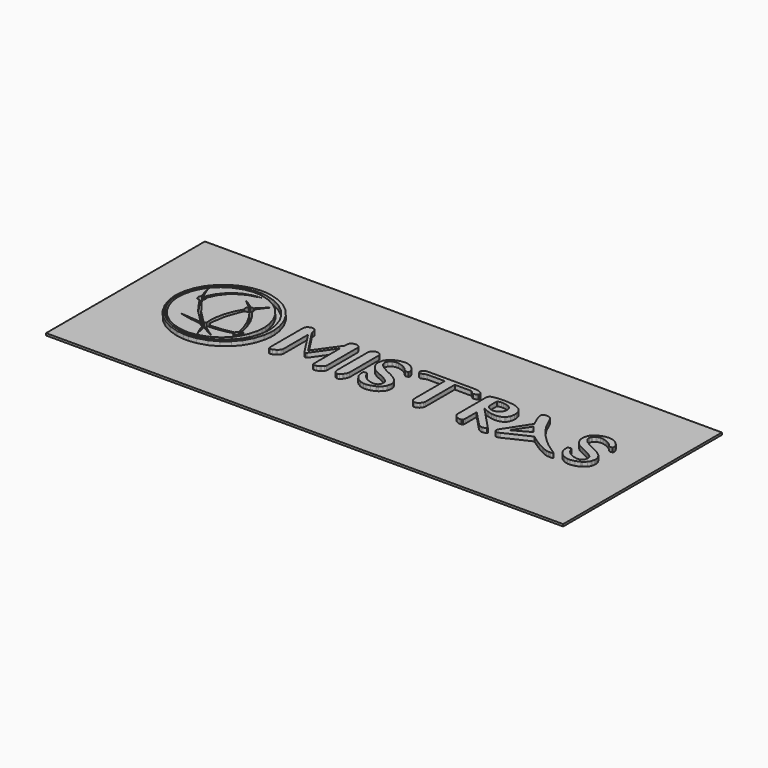
from build123d import *

# Parameters (mm, degrees)
F0_W     = 240
F0_H     = 92.1258560006
F1_DEPTH = 1
F2_DEPTH = 2


# Not quite as in the source:
# - a feature names something its author has since deleted; it is built from what else it names


with BuildPart() as f1:
    # F0 (on Top) → F1 (new body)
    with BuildSketch(Plane.XY):
        with Locations((5.0882510841, 17.9726510862)):
            Rectangle(F0_W, F0_H)
        Polygon((-73.0272497864, 43.6072834949), (-71.8914041604, 43.6072834949), (-70.7570980378, 43.6072834949), (-67.3526401667, 43.1595958993), (-63.1233163611, 41.871647335), (-59.2976503532, 39.8355001069), (-55.9637017388, 37.1392138106), (-53.21230122, 33.8705401414), (-51.1361269028, 30.1181544965), (-49.8229304824, 25.9722717765), (-49.3650821642, 22.6346283539), (-49.3650821642, 21.5206436765), (-49.3650821642, 20.4078906019), (-49.8229304824, 17.0702471793), (-51.1361269028, 12.9240565586), (-53.21230122, 9.1707472117), (-55.9637017388, 5.9014577411), (-59.2976503532, 3.2039398421), (-63.1233163611, 1.1674847133), (-67.3526401667, -0.120463851), (-70.7570980378, -0.5699988507), (-71.8914041604, -0.5699988507), (-73.0272497864, -0.5699988507), (-76.4317076575, -0.120463851), (-80.6597998604, 1.1674847133), (-84.4851579676, 3.2039398421), (-87.8194144826, 5.9014577411), (-90.5686596966, 9.1707472117), (-92.6469893186, 12.9240565586), (-93.9598778384, 17.0702471793), (-94.4161866531, 20.4078906019), (-94.4161866531, 21.5206436765), (-94.4161866531, 22.6346283539), (-93.9598778384, 25.9722717765), (-92.6469893186, 30.1181544965), (-90.5686596966, 33.8705401414), (-87.8194144826, 37.1392138106), (-84.4851579676, 39.8355001069), (-80.6597998604, 41.871647335), (-76.4317076575, 43.1595958993), align=None, mode=Mode.SUBTRACT)
        Polygon((-21.7975022568, 12.8058226957), (-21.7975022568, 26.0055250504), (-28.8401146188, 16.059717132), (-28.8903024305, 15.9861288684), (-29.4161968, 15.6169559474), (-29.592008091, 15.6169559474), (-29.7604297655, 15.6169559474), (-30.2232044947, 15.9744286423), (-30.2635394844, 16.0464774026), (-37.5900362777, 27.2552939298), (-37.5900362777, 12.9677784559), (-37.5900362777, 12.6952863499), (-37.9558222912, 11.8787337339), (-38.8062439825, 11.0433991762), (-39.0482539207, 10.8848303236), (-39.292111263, 10.7274930737), (-40.4181040671, 10.1745034439), (-41.3134792583, 9.9358804132), (-41.6109113197, 9.9358804132), (-41.7445402169, 9.9358804132), (-42.1337266824, 10.2179174405), (-42.1401925968, 10.2733395637), (-42.1469664119, 10.3299932897), (-42.2020806344, 11.1200664467), (-42.2057754427, 11.2222894741), (-42.2103939529, 11.3238967), (-42.2304074974, 12.5567310417), (-42.2304074974, 12.9659310518), (-42.2304074974, 30.1618763937), (-42.2304074974, 30.3786384758), (-42.0453591859, 31.0270773179), (-41.603829604, 31.626559951), (-41.4772824226, 31.7306303825), (-41.3519668439, 31.8340850126), (-40.6702747279, 32.1980236219), (-39.9836562009, 32.3535134677), (-39.753038588, 32.3535134677), (-39.5347370026, 32.3535134677), (-38.8749058352, 32.211571252), (-38.2849681232, 31.8790385125), (-38.1845925, 31.7838972009), (-38.0860642809, 31.6902953928), (-37.7402918119, 31.149005989), (-37.5900362777, 30.5710764038), (-37.5900362777, 30.3774068731), (-37.5900362777, 29.5137454524), (-29.8173913922, 17.5431826311), (-21.7975022568, 28.8101923877), (-21.7975022568, 30.0033075411), (-21.7975022568, 30.2200696231), (-21.6087591371, 30.8666610611), (-21.1675374558, 31.4661436943), (-21.0409902744, 31.5702141257), (-20.9156746957, 31.6736687558), (-20.2321351756, 32.0345283583), (-19.5424376418, 32.1897103034), (-19.3118200289, 32.1897103034), (-19.0947500462, 32.1897103034), (-18.4383057863, 32.0477680878), (-17.848675975, 31.7167748517), (-17.7498398552, 31.6219414408), (-17.6513116361, 31.5283396326), (-17.303691763, 30.9867423281), (-17.1518967255, 30.410660147), (-17.1518967255, 30.2169906163), (-17.1518967255, 12.8005883841), (-17.1518967255, 12.5385649013), (-17.5112168246, 11.7515707511), (-18.3480908857, 10.9611896934), (-18.5867139164, 10.8143210668), (-18.8256448477, 10.6692998443), (-19.9350110148, 10.1560294028), (-20.8254597951, 9.9358804132), (-21.1207365518, 9.9358804132), (-21.2260385859, 9.9358804132), (-21.5370182775, 10.0242479098), (-21.6955871302, 10.2296176665), (-21.7020530445, 10.2865792932), (-21.7106742637, 10.3450804233), (-21.7657884863, 11.0800393577), (-21.7691753938, 11.1687147549), (-21.7737939041, 11.2570822515), (-21.7975022568, 12.419715237), align=None, mode=Mode.SUBTRACT)
        Polygon((-7.3748183823, 30.405733736), (-7.3748183823, 30.2120642053), (-7.3748183823, 13.7476908903), (-7.3748183823, 13.447179822), (-7.6285285465, 12.544722915), (-8.2196978612, 11.4824655527), (-8.3871958337, 11.2601612583), (-8.5556175082, 11.0400122687), (-9.402652292, 10.2681052521), (-10.169324997, 9.9358804132), (-10.4248825653, 9.9358804132), (-10.6453394556, 9.9358804132), (-11.2281954518, 10.261331437), (-11.3017837154, 10.3266063822), (-11.3772193832, 10.3934208308), (-11.8615471603, 11.1853413919), (-11.8831002082, 11.2767878953), (-11.9065006603, 11.3688502), (-12.0167291054, 12.4431156891), (-12.0167291054, 12.8005883841), (-12.0167291054, 29.996533726), (-12.0167291054, 30.2136037088), (-11.8295254891, 30.859887246), (-11.3904591126, 31.4581382765), (-11.2632961298, 31.5615929066), (-11.1379805512, 31.6650475366), (-9.9356283772, 32.1829364884), (-9.534433785, 32.1829364884), (-9.3158242989, 32.1829364884), (-8.6578405356, 32.0425337761), (-8.0697502277, 31.7121563414), (-7.9709141079, 31.6167071291), (-7.8726937895, 31.5212579169), (-7.5247660157, 30.9821238179), align=None, mode=Mode.SUBTRACT)
        Polygon((-1.6315469098, 16.4085686078), (-1.6130728688, 16.3469884709), (-1.5465663209, 16.0698778546), (-0.8112994857, 14.7883952047), (0.4566355341, 13.6473152671), (0.7903998763, 13.4404060069), (1.1232405165, 13.2334967468), (2.7769750942, 12.5099301377), (4.2484324666, 12.1992583468), (4.7398419595, 12.1992583468), (5.164129103, 12.1992583468), (6.3279936913, 12.5733576787), (6.4419169447, 12.6487933465), (6.5539927939, 12.7236132129), (7.2052027422, 13.5925089452), (7.2236767832, 13.6910371643), (7.2403034202, 13.7911048869), (7.3671585023, 14.5260638213), (7.3739323174, 14.5744042288), (7.3803982318, 14.623052537), (7.412419903, 15.0639663176), (7.412419903, 15.2096033414), (7.412419903, 15.4032728721), (7.1867287011, 15.9827419608), (6.5170447118, 16.7728151179), (5.3978257227, 17.5798228126), (4.2333453331, 18.2177930313), (3.833998145, 18.4034571442), (3.4229507308, 18.5937397674), (2.1935032967, 19.1732088561), (0.8559827222, 19.8164133865), (-0.1779477772, 20.3343023382), (-0.7293979036, 20.6234210812), (-0.9098277048, 20.7234888038), (-1.1034972355, 20.835564653), (-2.0324336014, 21.5988504505), (-2.9077952481, 22.641402169), (-3.0749853199, 22.8901859223), (-3.2415595903, 23.1426644837), (-3.8250313879, 24.4352315583), (-4.0738151412, 25.6551340712), (-4.0738151412, 26.0609471737), (-4.0738151412, 26.29310429), (-3.9703605111, 26.9846492279), (-3.7261952681, 27.9917923677), (-3.655993912, 28.223949484), (-3.5857925559, 28.4576461037), (-2.8277410701, 29.5941075311), (-1.5247053722, 30.6914655715), (-1.1820119101, 30.9033012426), (-0.8396263487, 31.1172922185), (1.0410310337, 31.863951379), (2.9620234058, 32.1829364884), (3.6036884328, 32.1829364884), (4.0064225284, 32.1829364884), (5.2173959215, 31.9575531871), (6.4733228145, 31.4245771018), (6.7125616466, 31.2709346602), (6.9499530745, 31.120679126), (7.9133743171, 30.3740199655), (8.5719738817, 29.6387531304), (8.6588018748, 29.4934240072), (8.7437824638, 29.348094884), (9.0646149773, 28.7584650727), (9.2398104669, 28.3474176586), (9.2530501964, 28.2926113367), (9.2669057272, 28.2393445182), (9.3334122751, 27.854776563), (9.3334122751, 27.7260740768), (9.3334122751, 27.6207720426), (9.2881508744, 27.3304216969), (9.2801454566, 27.3036343373), (9.2696768333, 27.2783864812), (9.1813093368, 27.0582374916), (9.1729960183, 27.0397634505), (9.1046420663, 27.0280632245), (8.5984533406, 26.9276876012), (8.564892166, 26.9212216869), (8.531638892, 26.9144478718), (8.2843946422, 26.8827341013), (8.20249306, 26.8827341013), (8.0454637108, 26.8827341013), (7.6196370638, 27.0231368135), (7.5746835638, 27.0511557758), (7.5294221632, 27.0816379436), (7.1987368278, 27.3821490119), (6.7193354616, 27.8932641486), (6.6020253008, 28.0265851451), (6.4853309412, 28.1605219429), (5.6900234726, 28.8071133809), (4.6160658842, 29.4216831476), (4.3605083159, 29.5386854078), (4.1031033434, 29.6572271714), (2.0250816221, 30.2520912944), (1.3335366842, 30.2520912944), (0.8624486365, 30.2520912944), (-0.4104127942, 29.9112452364), (-0.5474285989, 29.8428912843), (-0.6844444036, 29.773921531), (-1.708522081, 28.8188136069), (-1.7753365296, 28.6950375316), (-1.8436904816, 28.5715693571), (-2.1829970362, 27.6943603062), (-2.1829970362, 27.4024704571), (-2.1829970362, 27.0462293649), (-1.7602493961, 25.9787376909), (-0.7746593042, 24.8779927429), (-0.4923143763, 24.6692360787), (-0.2118168525, 24.4604794144), (1.5755466224, 23.3646608774), (3.869098823, 22.2035673953), (4.4054618158, 21.9615574571), (4.9381300004, 21.7189317175), (7.1285354717, 20.5165795436), (8.6788154193, 19.3237722909), (8.894037998, 19.0848413596), (9.1077210732, 18.8477578323), (9.8562276378, 17.6063022715), (10.1767522506, 16.4187293304), (10.1767522506, 16.0227690498), (10.1767522506, 15.8290995191), (10.0785319321, 15.248090927), (9.8513012268, 14.2689667496), (9.7875657851, 14.0281884141), (9.7210592372, 13.7892574827), (8.9673183609, 12.6167716753), (7.6476560261, 11.4790786452), (7.2988045503, 11.2570822515), (6.9481056704, 11.0366253612), (5.0554401613, 10.2582524302), (3.1544613337, 9.9238722865), (2.5211096252, 9.9238722865), (1.9447195434, 9.9238722865), (0.2158571986, 10.3715598821), (-1.4794439716, 11.4125720973), (-1.7885762591, 11.709696258), (-2.0977085465, 12.0086678229), (-3.17843995, 13.5974353562), (-3.639367275, 15.1658814442), (-3.639367275, 15.6871573035), (-3.6495279976, 15.7573586596), (-3.6963289017, 16.1998119436), (-3.6963289017, 16.3469884709), (-3.6963289017, 16.4636828304), (-3.5928742716, 16.781436337), (-3.571013323, 16.8097632), (-3.5509997785, 16.838090063), (-3.1467261794, 17.0551600458), (-3.0848381418, 17.0702471793), (-3.0247975083, 17.0868738163), (-2.6553166866, 17.167235895), (-2.531848512, 17.167235895), (-2.3800534744, 17.167235895), (-1.9588453377, 16.9800322787), (-1.9237446597, 16.9418525938), (-1.8904913857, 16.9052124123), align=None, mode=Mode.SUBTRACT)
        Polygon((23.8383056324, 29.7843901542), (16.0034648086, 29.7843901542), (15.6044255212, 29.7843901542), (14.5554078882, 29.4250700552), (14.4082313609, 29.3514817915), (14.2576679261, 29.279740932), (13.6615722005, 29.0272623705), (13.3274999575, 28.9188813294), (13.2172715124, 28.9188813294), (13.0386891152, 28.9188813294), (12.5626746566, 29.1344118088), (12.5023261224, 29.1762863019), (12.4404380848, 29.2197002984), (12.1362322083, 29.7459025687), (12.1362322083, 29.9195585548), (12.1362322083, 30.0867486267), (12.3120434992, 30.5877030407), (12.7212435093, 31.0874258521), (12.8379378688, 31.1791802561), (12.9552480297, 31.2724741636), (13.681585745, 31.5966935846), (14.528312628, 31.7352488927), (14.8106575559, 31.7352488927), (36.1995944226, 31.7352488927), (36.5903203916, 31.7352488927), (37.7680405107, 31.5729852319), (38.8792540819, 31.1942673897), (39.0763105202, 31.085578448), (39.271827455, 30.9768895062), (39.9581380813, 30.4091206436), (40.2534148379, 29.8613653254), (40.2534148379, 29.677240716), (40.2534148379, 29.5251377777), (40.0498924853, 29.0657499561), (39.5757254308, 28.7353725213), (39.4417886329, 28.6916506241), (39.3066202323, 28.6485445282), (38.5350211164, 28.4311666448), (38.2773082433, 28.4311666448), (37.9537046236, 28.4311666448), (37.0817298844, 28.9973960041), (36.9813542612, 29.1094718533), (36.8828260421, 29.2227793053), (36.4616179054, 29.6153526783), (36.1829677857, 29.7843901542), (36.0909054809, 29.7843901542), (28.4802163556, 29.7843901542), (28.4802163556, 12.8005883841), (28.4802163556, 12.5518046308), (28.2514461468, 11.8032980662), (27.7169305581, 11.0095301009), (27.5651355205, 10.8561955599), (27.4111851781, 10.7025531182), (26.6260384321, 10.1661901254), (25.8913873983, 9.9358804132), (25.6472221553, 9.9358804132), (25.3965909979, 9.9358804132), (24.728446512, 10.2296176665), (24.6480844333, 10.2865792932), (24.5664907518, 10.3450804233), (24.0267408515, 11.1585540323), (24.0002613926, 11.2601612583), (23.9731661324, 11.3657711932), (23.8383056324, 12.4431156891), (23.8383056324, 12.8005883841), align=None, mode=Mode.SUBTRACT)
        Polygon((48.1165825248, 17.9471483295), (48.1165825248, 11.5308059602), (48.1165825248, 11.2419951179), (47.9946538536, 10.4251346013), (47.9712534016, 10.3715598821), (47.9463134461, 10.3182930637), (47.4718384909, 10.0008474577), (47.4016371348, 9.9909946358), (47.3314357787, 9.9823734166), (46.9256226762, 9.9358804132), (46.7904542756, 9.9358804132), (46.5031829367, 9.9358804132), (45.6459874304, 10.136323759), (44.7558465509, 10.602177495), (44.5868090749, 10.7358063922), (44.4183874004, 10.8694352894), (43.826910185, 11.5440456896), (43.5728921201, 12.1641576687), (43.5728921201, 12.3695274254), (43.5728921201, 29.3016018806), (43.5728921201, 29.4401571887), (43.6883548769, 29.8244172433), (43.7114474282, 29.8527441063), (43.7333083768, 29.8826104727), (44.2274889758, 30.3687856539), (44.304464147, 30.4356001025), (44.3798998148, 30.5039540545), (45.064363037, 30.8016940166), (46.1506366527, 31.0455513589), (46.427747269, 31.085578448), (46.7036262825, 31.1271450404), (49.404531089, 31.3294357903), (50.3063721946, 31.3294357903), (51.4773184987, 31.3294357903), (54.6148264762, 30.9787369103), (54.9843072979, 30.9069960508), (55.3537881196, 30.8383341981), (57.0041357898, 30.2567098046), (58.3958468848, 29.3616425141), (58.6360094189, 29.1359513122), (58.8730929461, 28.910568011), (59.7105828086, 27.5591919056), (60.0677476029, 26.0424731326), (60.0677476029, 25.5362844069), (60.0677476029, 24.9183277326), (59.7105828086, 23.0604550009), (58.8730929461, 21.62563781), (58.6360094189, 21.4218075567), (58.3958468848, 21.2195168069), (56.9856617487, 20.5098057285), (55.4215262702, 20.205599852), (54.901174113, 20.205599852), (54.4116120243, 20.205599852), (52.9490837718, 20.3860296533), (51.2639433242, 20.8056982866), (50.9197103586, 20.9239321495), (50.5739378897, 21.0443213172), (49.232722507, 21.5936161388), (48.3989274527, 22.0764044125), (48.3087125521, 22.1620008029), (57.4136437005, 12.5299436822), (57.6507272277, 12.2826994323), (58.5282441792, 11.3439102446), (58.9900952063, 10.8093946558), (59.0208852748, 10.7607463477), (59.0485963364, 10.7142533443), (59.017806268, 10.4085079643), (58.9839371926, 10.3949603342), (58.8299868503, 10.3198325671), (57.5060139059, 9.9358804132), (57.0657159267, 9.9358804132), (56.797842331, 9.9358804132), (56.0650387013, 10.0830569405), (55.9849845233, 10.1110759029), (55.9049303452, 10.14125017), (55.0951515444, 10.6723788511), (55.0150973663, 10.7490461216), align=None, mode=Mode.SUBTRACT)
        Polygon((70.6071880415, 31.6099333141), (70.7026372538, 31.5966935846), (70.8781406441, 31.574832636), (71.706393486, 31.0286168213), (72.4761451979, 29.9078583288), (72.6177795129, 29.5968786372), (72.7624928347, 29.286514747), (74.3173912926, 25.9288577799), (74.4836576624, 25.5676902767), (74.7915583471, 24.9999214141), (76.5958563597, 22.2386680734), (78.7665561871, 19.5796377599), (79.2561182758, 19.0632883116), (79.7426013577, 18.5469388633), (82.0210664248, 16.2986480634), (84.0809220057, 14.4928105474), (84.4596398479, 14.19722589), (84.8352786833, 13.901333332), (86.6180236479, 12.5816709972), (88.2529762839, 11.4692258232), (88.5577979618, 11.2767878953), (88.7363803589, 11.1634804433), (89.2813645709, 10.8177079743), (89.6847144679, 10.5421368615), (89.8632968651, 10.385415413), (89.9033239541, 10.3032059301), (89.9033239541, 10.2748790671), (89.9033239541, 10.2216122487), (89.6662404269, 10.0812095364), (89.6200553241, 10.0578090844), (89.5707912146, 10.0359481358), (88.9057257355, 9.9207932797), (88.6840372425, 9.9207932797), (88.4592697427, 9.9207932797), (87.7849672431, 9.9577413619), (86.8366331341, 10.1095363994), (85.7559017307, 10.4451481458), (84.7675405327, 10.8728221969), (84.4473238205, 11.0347779571), (83.9639197455, 11.2804827035), (81.774745877, 12.476368963), (79.8965517001, 13.6260701198), (79.5670979674, 13.8477586128), (79.2376442347, 14.0719103113), (77.7905110165, 15.0673532251), (76.6020143734, 15.9079220944), (76.4049579352, 16.0514038135), (64.969526504, 10.6455914916), (64.8987093465, 10.6104908135), (64.2675129427, 10.3383066082), (64.2120908195, 10.3198325671), (64.1597477031, 10.3032059301), (63.7317657513, 10.2129910295), (63.5932104432, 10.2129910295), (63.3899959912, 10.2129910295), (62.8480907861, 10.4719355054), (62.7926686629, 10.5239707211), (62.7341675327, 10.5772375396), (62.4570569165, 11.1366930837), (62.4570569165, 11.3223571966), (62.4570569165, 11.5160267273), (62.5925332178, 12.027141864), (62.6202442794, 12.0924168092), (62.647955341, 12.1573838536), (63.0297521901, 12.8689423361), (63.0790162997, 12.9459175072), (70.1884431103, 23.7840216101), (70.0468087953, 24.0996198119), (68.7074408167, 27.2201932517), (68.5812015359, 27.5290176385), (68.4518832483, 27.838149926), (68.0023482486, 29.1325644047), (67.8114498241, 29.968206863), (67.8114498241, 30.2453174793), (67.8114498241, 30.5159621812), (68.1686146184, 31.2690872561), (68.2394317759, 31.3260488827), (68.3133279402, 31.3860895163), (68.8152060563, 31.591459273), (69.4587184874, 31.6801346702), (69.6742489668, 31.6801346702), (69.9298065351, 31.6801346702), align=None, mode=Mode.SUBTRACT)
        Polygon((93.1516761781, 16.4085686078), (93.1701502192, 16.3469884709), (93.2378883698, 16.0698778546), (93.9768500132, 14.7868557013), (95.2423218275, 13.6460836643), (95.5779335738, 13.4385586028), (95.9104663134, 13.2316493427), (97.5638929904, 12.5080827336), (99.0356582635, 12.1977188433), (99.5252203522, 12.1977188433), (99.9501232971, 12.1977188433), (101.1170668923, 12.5718181753), (101.2279111388, 12.6454064389), (101.3418343921, 12.7217658088), (101.9945838438, 13.5909694418), (102.0130578849, 13.6891897602), (102.031531926, 13.7892574827), (102.151613193, 14.5245243179), (102.1577712067, 14.5731726261), (102.1639292204, 14.6215130336), (102.2008773026, 15.06057941), (102.2008773026, 15.2059085332), (102.2008773026, 15.3998859646), (101.9730307959, 15.9808945567), (101.3018073031, 16.7712756144), (100.1841278175, 17.5782833091), (99.0202632292, 18.2144061238), (98.6199923391, 18.4000702367), (98.2104844284, 18.5903528599), (96.9788816894, 19.1701298492), (95.6425927176, 19.8148738831), (94.6049674101, 20.3327628348), (94.0538251844, 20.6234210812), (93.8752427872, 20.7234888038), (93.6812653558, 20.835564653), (92.7514052879, 21.5970030464), (91.8769673433, 22.6398626656), (91.7107009735, 22.8901859223), (91.5444346038, 23.1426644837), (90.9594233028, 24.4352315583), (90.7100237481, 25.6551340712), (90.7100237481, 26.0609471737), (90.7100237481, 26.2912568859), (90.8147099809, 26.9828018238), (91.0610305287, 27.9917923677), (91.1318476862, 28.223949484), (91.2026648437, 28.4576461037), (91.9570215213, 29.5941075311), (93.2625204246, 30.6914655715), (93.6042901847, 30.9033012426), (93.9460599447, 31.1172922185), (95.8273331285, 31.863951379), (97.7486334012, 32.1829364884), (98.3890668255, 32.1829364884), (98.7924167225, 32.1829364884), (100.0055454204, 31.9575531871), (101.2587012073, 31.4245771018), (101.4988637414, 31.2709346602), (101.7359472686, 31.120679126), (102.6996764118, 30.3740199655), (103.3585838772, 29.6387531304), (103.4447960689, 29.4934240072), (103.5310082606, 29.348094884), (103.8512249728, 28.7584650727), (104.0267283631, 28.3474176586), (104.0421233973, 28.2926113367), (104.0544394247, 28.2393445182), (104.1221775753, 27.8532370596), (104.1221775753, 27.7229950699), (104.1221775753, 27.6192325392), (104.0729134658, 27.3304216969), (104.0667554521, 27.3036343373), (104.0544394247, 27.2771548784), (103.968227233, 27.0582374916), (103.9589902124, 27.0397634505), (103.8912520618, 27.026523721), (103.3862949388, 26.9276876012), (103.3524258635, 26.9212216869), (103.3185567882, 26.9144478718), (103.0691572335, 26.8811945978), (102.9860240487, 26.8811945978), (102.8289946994, 26.8811945978), (102.4071707613, 27.0231368135), (102.3640646655, 27.0511557758), (102.3178795628, 27.0816379436), (101.9853468233, 27.3821490119), (101.5081007619, 27.8932641486), (101.3910985017, 28.0265851451), (101.2740962415, 28.1605219429), (100.476633468, 28.8071133809), (99.4020600783, 29.4216831476), (99.14650251, 29.5386854078), (98.8909449416, 29.6572271714), (96.8095363128, 30.2487043868), (96.119838779, 30.2487043868), (95.6487507313, 30.2487043868), (94.3771209034, 29.9112452364), (94.2416446021, 29.8428912843), (94.1030892939, 29.773921531), (93.0808590206, 28.8188136069), (93.01312087, 28.6950375316), (92.9453827193, 28.5715693571), (92.6036129593, 27.6943603062), (92.6036129593, 27.400623053), (92.6036129593, 27.0446898614), (93.0285159042, 25.9768902868), (94.0137980954, 24.8761453388), (94.2939877185, 24.6676965753), (94.5772563484, 24.458939911), (96.3630803199, 23.3646608774), (98.6569404212, 22.2035673953), (99.1926876127, 21.9615574571), (99.7253557973, 21.7189317175), (101.9145296658, 20.5147321395), (103.4663491168, 19.3203853834), (103.6818795962, 19.081454452), (103.8943310686, 18.8443709248), (104.6394507257, 17.604762768), (104.9627464447, 16.417189827), (104.9627464447, 16.0212295464), (104.9627464447, 15.8275600157), (104.8642182256, 15.2462435229), (104.6363717189, 14.2674272461), (104.5747915819, 14.0281884141), (104.5070534313, 13.7892574827), (103.7526967537, 12.6149242712), (102.434881823, 11.4775391417), (102.0869540492, 11.255542748), (101.7359472686, 11.0332384537), (99.8423580575, 10.2548655226), (97.9426108326, 9.9207932797), (97.3114144289, 9.9207932797), (96.7325611416, 9.9207932797), (95.0021592934, 10.3681729746), (93.3056265205, 11.4107246931), (92.9946468289, 11.7063093505), (92.6867461441, 12.0055888161), (91.6060147407, 13.5937405479), (91.1441637136, 15.1624945367), (91.1441637136, 15.6837703959), (91.1349266931, 15.7555112555), (91.0918205972, 16.1998119436), (91.0918205972, 16.3469884709), (91.0918205972, 16.462143327), (91.1934278232, 16.7780494295), (91.2149808711, 16.8063762925), (91.2334549122, 16.8350110562), (91.6368048092, 17.0551600458), (91.6983849461, 17.0702471793), (91.7599650831, 17.0868738163), (92.1294459048, 17.1638489875), (92.2526061787, 17.1638489875), (92.4034775142, 17.1638489875), (92.8253014523, 16.9784927753), (92.8591705276, 16.9400051897), (92.8930396029, 16.9033650082), align=None, mode=Mode.SUBTRACT)
        Polygon((-70.7570980378, 43.6072834949), (-71.8914041604, 43.6072834949), (-73.0272497864, 43.6072834949), (-76.4317076575, 43.1595958993), (-80.6597998604, 41.871647335), (-84.4851579676, 39.8355001069), (-87.8194144826, 37.1392138106), (-90.5686596966, 33.8705401414), (-92.6469893186, 30.1181544965), (-93.9598778384, 25.9722717765), (-94.4161866531, 22.6346283539), (-94.4161866531, 21.5206436765), (-94.4161866531, 20.4078906019), (-93.9598778384, 17.0702471793), (-92.6469893186, 12.9240565586), (-90.5686596966, 9.1707472117), (-87.8194144826, 5.9014577411), (-84.4851579676, 3.2039398421), (-80.6597998604, 1.1674847133), (-76.4317076575, -0.120463851), (-73.0272497864, -0.5699988507), (-71.8914041604, -0.5699988507), (-70.7570980378, -0.5699988507), (-67.3526401667, -0.120463851), (-63.1233163611, 1.1674847133), (-59.2976503532, 3.2039398421), (-55.9637017388, 5.9014577411), (-53.21230122, 9.1707472117), (-51.1361269028, 12.9240565586), (-49.8229304824, 17.0702471793), (-49.3650821642, 20.4078906019), (-49.3650821642, 21.5206436765), (-49.3650821642, 22.6346283539), (-49.8229304824, 25.9722717765), (-51.1361269028, 30.1181544965), (-53.21230122, 33.8705401414), (-55.9637017388, 37.1392138106), (-59.2976503532, 39.8355001069), (-63.1233163611, 41.871647335), (-67.3526401667, 43.1595958993), align=None)
        Polygon((-71.2466601265, 0.5242801828), (-72.3255441259, 0.5242801828), (-73.40658343, 0.5242801828), (-76.6472381369, 0.9467199223), (-80.6696526823, 2.1580012161), (-84.3115019814, 4.0740671772), (-87.4838027362, 6.6114767201), (-90.0997269538, 9.6867887593), (-92.0758335484, 13.2165622091), (-93.3252945271, 17.1170480834), (-93.7594344926, 20.2573271671), (-93.7594344926, 21.3032657931), (-93.7594344926, 22.3507439226), (-93.3252945271, 25.4913309069), (-92.0758335484, 29.3899693771), (-90.0997269538, 32.9178954228), (-87.4838027362, 35.993207462), (-84.3115019814, 38.5309249056), (-80.6696526823, 40.4454513633), (-76.6472381369, 41.6564247564), (-73.40658343, 42.0773249924), (-72.3255441259, 42.0773249924), (-71.2466601265, 42.0773249924), (-68.0078528238, 41.6564247564), (-63.984822477, 40.4454513633), (-60.3435889793, 38.5309249056), (-57.1731356285, 35.993207462), (-54.5553640069, 32.9178954228), (-52.5792574122, 29.3899693771), (-51.3297964335, 25.4913309069), (-50.8935011633, 22.3507439226), (-50.8935011633, 21.3032657931), (-50.8935011633, 20.2573271671), (-51.3297964335, 17.1170480834), (-52.5792574122, 13.2165622091), (-54.5553640069, 9.6867887593), (-57.1731356285, 6.6114767201), (-60.3435889793, 4.0740671772), (-63.984822477, 2.1580012161), (-68.0078528238, 0.9467199223), align=None, mode=Mode.SUBTRACT)
        Polygon((-73.40658343, 0.5242801828), (-72.3255441259, 0.5242801828), (-71.2466601265, 0.5242801828), (-68.0078528238, 0.9467199223), (-63.984822477, 2.1580012161), (-60.3435889793, 4.0740671772), (-57.1731356285, 6.6114767201), (-54.5553640069, 9.6867887593), (-52.5792574122, 13.2165622091), (-51.3297964335, 17.1170480834), (-50.8935011633, 20.2573271671), (-50.8935011633, 21.3032657931), (-50.8935011633, 22.3507439226), (-51.3297964335, 25.4913309069), (-52.5792574122, 29.3899693771), (-54.5553640069, 32.9178954228), (-57.1731356285, 35.993207462), (-60.3435889793, 38.5309249056), (-63.984822477, 40.4454513633), (-68.0078528238, 41.6564247564), (-71.2466601265, 42.0773249924), (-72.3255441259, 42.0773249924), (-73.40658343, 42.0773249924), (-76.6472381369, 41.6564247564), (-80.6696526823, 40.4454513633), (-84.3115019814, 38.5309249056), (-87.4838027362, 35.993207462), (-90.0997269538, 32.9178954228), (-92.0758335484, 29.3899693771), (-93.3252945271, 25.4913309069), (-93.7594344926, 22.3507439226), (-93.7594344926, 21.3032657931), (-93.7594344926, 20.2573271671), (-93.3252945271, 17.1170480834), (-92.0758335484, 13.2165622091), (-90.0997269538, 9.6867887593), (-87.4838027362, 6.6114767201), (-84.3115019814, 4.0740671772), (-80.6696526823, 2.1580012161), (-76.6472381369, 0.9467199223), align=None)
        Polygon((-59.2175961752, 10.5756980361), (-59.1009018157, 10.573850632), (-59.0337794664, 10.5720032279), (-58.2905072134, 10.7807598922), (-58.2116846381, 10.8192474778), (-58.1969054053, 10.6372781731), (-58.1267040491, 8.8000347872), (-58.1267040491, 8.6143706743), (-58.799774946, 7.8193711063), (-61.1536756808, 5.7176410323), (-64.7401028566, 3.5127642289), (-68.7809914432, 2.1096608086), (-72.0733734651, 1.617019713), (-73.1691920021, 1.617019713), (-74.161555909, 1.617019713), (-77.1364923249, 2.0175985038), (-80.8319163431, 3.1654522565), (-84.1760256801, 4.979603091), (-87.0893819591, 7.3833837368), (-89.4931626048, 10.2979716185), (-91.3073134393, 13.6426967568), (-92.455167192, 17.3375049737), (-92.8538985788, 20.3124413896), (-92.8538985788, 21.3032657931), (-92.8538985788, 22.1435267618), (-92.568474644, 24.6590753561), (-91.7433008089, 27.8282971041), (-90.426717481, 30.7665933386), (-89.1575508585, 32.8027405667), (-88.6661413656, 33.4274710561), (-88.5509865095, 32.8612416968), (-87.8027878456, 30.0947540445), (-86.8421377092, 27.41724969), (-86.6198334149, 26.8944343273), (-86.7402225826, 26.770658252), (-87.1177088221, 26.0107593621), (-87.1561964077, 25.1686509893), (-87.1044690926, 25.004847825), (-87.0625945995, 24.868139921), (-86.8255110723, 24.4835719658), (-86.3929106102, 24.1445733119), (-85.861781929, 24.0078654079), (-85.417481241, 24.0463529935), (-85.281697039, 24.0928459968), (-84.6036997312, 22.8098238435), (-80.3839208469, 16.9052124123), (-75.2425952131, 11.7297098025), (-74.1015152754, 10.8127815634), (-74.9587107818, 10.839568923), (-83.4995678757, 11.5526669088), (-84.3447552553, 11.6665901622), (-83.4195136977, 11.3790109226), (-78.7671343513, 10.3266063822), (-74.1917301761, 9.7502163003), (-73.3028208992, 9.7003363894), (-73.2729545328, 9.5414596361), (-72.8320407523, 8.9081079276), (-72.1352615027, 8.5943571298), (-71.9031043864, 8.5943571298), (-71.8529165748, 8.5943571298), (-71.6977346297, 8.6143706743), (-71.6777210852, 8.6162180785), (-71.5437842873, 8.0598415411), (-71.0258953356, 6.4141123812), (-70.3460506237, 4.7455985706), (-69.7816686686, 3.6263795816), (-69.5144108742, 3.1586784415), (-69.4676099701, 3.0666161367), (-69.6160181002, 3.4961375919), (-70.6333219625, 7.8624772022), (-70.6902835892, 8.3033909828), (-70.1489941854, 7.9394523734), (-67.3628008892, 6.2441512032), (-64.4947060109, 4.7271245295), (-63.9100026106, 4.4518613174), (-64.5011719253, 4.8225737418), (-70.0575476821, 8.7529259825), (-70.5751287331, 9.1621259925), (-70.5403359558, 9.1972266706), (-70.2407485895, 9.5950343552), (-70.2176560381, 9.6381404511), (-69.6212524118, 9.6467616703), (-66.7679367663, 9.8253440674), (-64.1353859118, 10.1760429473), (-63.6476712272, 10.2714921596), (-63.2784983062, 10.3364592041), (-61.5795023278, 10.7290325771), (-60.0729442774, 11.1936547104), (-59.798912668, 11.2921829295), (-59.8022995755, 11.1853413919), (-59.6286435893, 10.7742939778), align=None, mode=Mode.SUBTRACT)
        Polygon((-70.0138257848, 10.7875337072), (-70.0603187882, 10.7859942038), (-70.0889535519, 10.8946831455), (-70.3694510757, 11.3488366555), (-70.805746346, 11.6681296656), (-70.9125878836, 11.7063093505), (-70.9209012021, 13.0564538531), (-69.8817363911, 19.744672527), (-67.568170646, 26.1659413072), (-66.9369742423, 27.3806095085), (-66.9034130676, 27.3738356934), (-66.6244550472, 27.3316532996), (-66.5191530131, 27.3316532996), (-66.2300342701, 27.3316532996), (-65.3614464384, 27.7279214809), (-65.2764658495, 27.7978149363), (-64.6366482266, 27.0111286868), (-62.9025515701, 24.4974274966), (-60.953232335, 20.9442535947), (-59.4762327503, 17.1890968436), (-58.6917018056, 14.270506253), (-58.5208169256, 13.2815292536), (-58.6147266344, 13.2116357982), (-59.4146526134, 12.3378136549), (-59.4750011476, 12.2377459324), (-59.4848539695, 12.2211192954), (-59.5682950551, 12.0607030386), (-59.5769162743, 12.043768501), (-60.3700684381, 11.8266985182), (-64.4780793739, 11.1382325871), (-68.6556758645, 10.8244817894), (-69.4842366071, 10.7927680189), (-69.5325770146, 10.7927680189), align=None, mode=Mode.SUBTRACT)
        Polygon((-74.3050376281, 40.9830459589), (-73.1691920021, 40.9830459589), (-72.1789833999, 40.9830459589), (-69.2037390833, 40.5840066715), (-65.5086229658, 39.4361529188), (-62.1660531322, 37.6220020843), (-59.2526968532, 35.2182214385), (-56.8489162075, 32.3064046629), (-55.034765373, 28.9641427301), (-53.887219521, 25.2687187119), (-53.4863328294, 22.2953217993), (-53.4863328294, 21.3032657931), (-53.4863328294, 20.4377569683), (-53.7917703087, 17.8387672884), (-54.6686714588, 14.571325222), (-56.069003773, 11.5545143129), (-57.4151455667, 9.4749530882), (-57.9345740219, 8.8397539756), (-57.9093261657, 9.0306524001), (-57.7541442206, 10.9211626044), (-57.7492178096, 11.1083662207), (-57.6506895905, 11.1819544844), (-56.7971888924, 12.0942642133), (-56.7316060466, 12.1992583468), (-56.6952737658, 12.2626858878), (-56.4563428344, 12.8443102813), (-56.4446426084, 12.8975770997), (-56.2355780435, 13.0278190894), (-55.5073929241, 13.5404737295), (-55.2201215852, 13.7827915684), (-55.3186498043, 13.7295247499), (-56.3159401222, 13.2316493427), (-56.4160078447, 13.1845405379), (-56.4193947523, 13.2867635653), (-56.6001324542, 13.6741026267), (-57.000711245, 13.8628457464), (-57.1127870943, 13.8646931505), (-57.169748721, 13.8662326539), (-57.7760051692, 13.7190561266), (-57.8394327103, 13.6910371643), (-57.9478137513, 14.803790239), (-58.6997072234, 18.0977117643), (-60.2567609862, 22.1435267618), (-62.2898292075, 25.6597525815), (-63.9481822955, 27.8282971041), (-64.5781470965, 28.4745806414), (-64.5895394218, 28.4862808674), (-64.7016152711, 28.5980488159), (-64.7117759936, 28.6100569427), (-64.6936098532, 28.6617842577), (-64.5895394218, 29.1026980382), (-64.5895394218, 29.2665012025), (-64.5895394218, 29.4435440962), (-64.7268631272, 29.9712858699), (-65.0172134729, 30.4740876881), (-65.0941886441, 30.559068277), (-64.8389389764, 30.9568759617), (-62.0173371015, 34.7021798909), (-61.7097443174, 35.0510313667), (-62.1060124987, 34.7619126237), (-63.9451032886, 33.1854611179), (-65.6068432842, 31.4562908724), (-65.9144360682, 31.0920443623), (-65.9627764757, 31.1086709993), (-66.3688974789, 31.1976542972), (-66.5191530131, 31.1976542972), (-66.6995828143, 31.1976542972), (-67.2393327147, 31.0587910884), (-67.2978338448, 31.0320037288), (-67.7538347589, 31.4113373724), (-69.1837255388, 32.4754421389), (-70.7453978118, 33.4893590937), (-71.87323802, 34.1205554974), (-72.3640317115, 34.3730340589), (-72.4560940162, 34.4229139698), (-72.0484335096, 34.1439559495), (-68.2261544093, 30.9953635473), (-67.8705291184, 30.6458962701), (-67.960744019, 30.559068277), (-68.2963557654, 30.0279395959), (-68.4521535119, 29.4567838257), (-68.4521535119, 29.2665012025), (-68.4521535119, 29.0041698191), (-68.1393264162, 28.2156361655), (-68.0811331867, 28.1352740868), (-68.642436135, 27.2500596182), (-70.0655530999, 24.4238392329), (-71.4354032463, 20.6249605846), (-72.1903757253, 16.9199916452), (-72.3726529306, 14.3357811982), (-72.3255441259, 13.4788935925), (-72.3209256156, 13.3184773358), (-72.2088497664, 11.7814371176), (-72.1922231294, 11.6330289875), (-72.2624244855, 11.6028547204), (-72.8652940262, 11.1487012104), (-72.9136344337, 11.0898921796), (-74.0547143714, 12.0739427681), (-79.0442449676, 17.0970345389), (-82.9884527391, 22.0850256317), (-83.6064094133, 23.0490626756), (-83.6913900023, 23.1793046652), (-84.4799236559, 24.4503186918), (-84.5535119196, 24.5740947671), (-84.4414360703, 24.6975629417), (-84.0827317726, 25.4494564138), (-84.0507101014, 26.2712433414), (-84.0993584096, 26.429812194), (-84.112598139, 26.4716866871), (-84.3013412588, 26.832238389), (-84.3228943067, 26.8642600602), (-84.1344590877, 27.5708921317), (-82.5336834277, 31.0052163692), (-80.0867966861, 34.0854548194), (-79.4737664228, 34.6135044937), (-78.7154070363, 35.2951966097), (-74.2268308541, 37.827371841), (-69.1470853573, 39.2458702956), (-68.0928334128, 39.3677989667), (-68.2797291284, 39.3591777476), (-69.0032957375, 39.3228454668), (-70.5517282811, 39.1522684874), (-72.6497635469, 38.7412210733), (-74.5793771382, 38.1934657551), (-75.2056471309, 37.9662350498), (-75.9556931989, 37.7072905739), (-78.0888291428, 36.5846846774), (-81.0138856478, 34.3496336069), (-83.5860879681, 31.2909482047), (-85.0984961316, 28.4410194667), (-85.4122469293, 27.4323368235), (-85.4639742444, 27.4338763269), (-85.9951029255, 27.3218004777), (-86.0468302406, 27.2968605222), (-86.3060826171, 27.809823063), (-87.0274939215, 29.371495336), (-87.7590659484, 31.1406926705), (-88.2720284892, 32.5422565874), (-88.5177332356, 33.2738286144), (-88.5959400095, 33.5176859567), (-87.9262560202, 34.363181237), (-85.5440284224, 36.6031587185), (-81.8756996644, 38.9549041485), (-77.7113429033, 40.4568436887), align=None, mode=Mode.SUBTRACT)
        Polygon((-72.1789833999, 40.9830459589), (-73.1691920021, 40.9830459589), (-74.3050376281, 40.9830459589), (-77.7113429033, 40.4568436887), (-81.8756996644, 38.9549041485), (-85.5440284224, 36.6031587185), (-87.9262560202, 34.363181237), (-88.5959400095, 33.5176859567), (-88.5177332356, 33.2738286144), (-88.2720284892, 32.5422565874), (-87.7590659484, 31.1406926705), (-87.0274939215, 29.371495336), (-86.3060826171, 27.809823063), (-86.0468302406, 27.2968605222), (-85.9951029255, 27.3218004777), (-85.4639742444, 27.4338763269), (-85.4122469293, 27.4323368235), (-85.0984961316, 28.4410194667), (-83.5860879681, 31.2909482047), (-81.0138856478, 34.3496336069), (-78.0888291428, 36.5846846774), (-75.9556931989, 37.7072905739), (-75.2056471309, 37.9662350498), (-74.5793771382, 38.1934657551), (-72.6497635469, 38.7412210733), (-70.5517282811, 39.1522684874), (-69.0032957375, 39.3228454668), (-68.2797291284, 39.3591777476), (-68.0928334128, 39.3677989667), (-69.1470853573, 39.2458702956), (-74.2268308541, 37.827371841), (-78.7154070363, 35.2951966097), (-79.4737664228, 34.6135044937), (-80.0867966861, 34.0854548194), (-82.5336834277, 31.0052163692), (-84.1344590877, 27.5708921317), (-84.3228943067, 26.8642600602), (-84.3013412588, 26.832238389), (-84.112598139, 26.4716866871), (-84.0993584096, 26.429812194), (-84.0507101014, 26.2712433414), (-84.0827317726, 25.4494564138), (-84.4414360703, 24.6975629417), (-84.5535119196, 24.5740947671), (-84.4799236559, 24.4503186918), (-83.6913900023, 23.1793046652), (-83.6064094133, 23.0490626756), (-82.9884527391, 22.0850256317), (-79.0442449676, 17.0970345389), (-74.0547143714, 12.0739427681), (-72.9136344337, 11.0898921796), (-72.8652940262, 11.1487012104), (-72.2624244855, 11.6028547204), (-72.1922231294, 11.6330289875), (-72.2088497664, 11.7814371176), (-72.3209256156, 13.3184773358), (-72.3255441259, 13.4788935925), (-72.3726529306, 14.3357811982), (-72.1903757253, 16.9199916452), (-71.4354032463, 20.6249605846), (-70.0655530999, 24.4238392329), (-68.642436135, 27.2500596182), (-68.0811331867, 28.1352740868), (-68.1393264162, 28.2156361655), (-68.4521535119, 29.0041698191), (-68.4521535119, 29.2665012025), (-68.4521535119, 29.4567838257), (-68.2963557654, 30.0279395959), (-67.960744019, 30.559068277), (-67.8705291184, 30.6458962701), (-68.2261544093, 30.9953635473), (-72.0484335096, 34.1439559495), (-72.4560940162, 34.4229139698), (-72.3640317115, 34.3730340589), (-71.87323802, 34.1205554974), (-70.7453978118, 33.4893590937), (-69.1837255388, 32.4754421389), (-67.7538347589, 31.4113373724), (-67.2978338448, 31.0320037288), (-67.2393327147, 31.0587910884), (-66.6995828143, 31.1976542972), (-66.5191530131, 31.1976542972), (-66.3688974789, 31.1976542972), (-65.9627764757, 31.1086709993), (-65.9144360682, 31.0920443623), (-65.6068432842, 31.4562908724), (-63.9451032886, 33.1854611179), (-62.1060124987, 34.7619126237), (-61.7097443174, 35.0510313667), (-62.0173371015, 34.7021798909), (-64.8389389764, 30.9568759617), (-65.0941886441, 30.559068277), (-65.0172134729, 30.4740876881), (-64.7268631272, 29.9712858699), (-64.5895394218, 29.4435440962), (-64.5895394218, 29.2665012025), (-64.5895394218, 29.1026980382), (-64.6936098532, 28.6617842577), (-64.7117759936, 28.6100569427), (-64.7016152711, 28.5980488159), (-64.5895394218, 28.4862808674), (-64.5781470965, 28.4745806414), (-63.9481822955, 27.8282971041), (-62.2898292075, 25.6597525815), (-60.2567609862, 22.1435267618), (-58.6997072234, 18.0977117643), (-57.9478137513, 14.803790239), (-57.8394327103, 13.6910371643), (-57.7760051692, 13.7190561266), (-57.169748721, 13.8662326539), (-57.1127870943, 13.8646931505), (-57.000711245, 13.8628457464), (-56.6001324542, 13.6741026267), (-56.4193947523, 13.2867635653), (-56.4160078447, 13.1845405379), (-56.3159401222, 13.2316493427), (-55.3186498043, 13.7295247499), (-55.2201215852, 13.7827915684), (-55.5073929241, 13.5404737295), (-56.2355780435, 13.0278190894), (-56.4446426084, 12.8975770997), (-56.4563428344, 12.8443102813), (-56.6952737658, 12.2626858878), (-56.7316060466, 12.1992583468), (-56.7971888924, 12.0942642133), (-57.6506895905, 11.1819544844), (-57.7492178096, 11.1083662207), (-57.7541442206, 10.9211626044), (-57.9093261657, 9.0306524001), (-57.9345740219, 8.8397539756), (-57.4151455667, 9.4749530882), (-56.069003773, 11.5545143129), (-54.6686714588, 14.571325222), (-53.7917703087, 17.8387672884), (-53.4863328294, 20.4377569683), (-53.4863328294, 21.3032657931), (-53.4863328294, 22.2953217993), (-53.887219521, 25.2687187119), (-55.034765373, 28.9641427301), (-56.8489162075, 32.3064046629), (-59.2526968532, 35.2182214385), (-62.1660531322, 37.6220020843), (-65.5086229658, 39.4361529188), (-69.2037390833, 40.5840066715), align=None)
        Polygon((-59.0337794664, 10.5720032279), (-59.1009018157, 10.573850632), (-59.2175961752, 10.5756980361), (-59.6286435893, 10.7742939778), (-59.8022995755, 11.1853413919), (-59.798912668, 11.2921829295), (-60.0729442774, 11.1936547104), (-61.5795023278, 10.7290325771), (-63.2784983062, 10.3364592041), (-63.6476712272, 10.2714921596), (-64.1353859118, 10.1760429473), (-66.7679367663, 9.8253440674), (-69.6212524118, 9.6467616703), (-70.2176560381, 9.6381404511), (-70.2407485895, 9.5950343552), (-70.5403359558, 9.1972266706), (-70.5751287331, 9.1621259925), (-70.0575476821, 8.7529259825), (-64.5011719253, 4.8225737418), (-63.9100026106, 4.4518613174), (-64.4947060109, 4.7271245295), (-67.3628008892, 6.2441512032), (-70.1489941854, 7.9394523734), (-70.6902835892, 8.3033909828), (-70.6333219625, 7.8624772022), (-69.6160181002, 3.4961375919), (-69.4676099701, 3.0666161367), (-69.5144108742, 3.1586784415), (-69.7816686686, 3.6263795816), (-70.3460506237, 4.7455985706), (-71.0258953356, 6.4141123812), (-71.5437842873, 8.0598415411), (-71.6777210852, 8.6162180785), (-71.6977346297, 8.6143706743), (-71.8529165748, 8.5943571298), (-71.9031043864, 8.5943571298), (-72.1352615027, 8.5943571298), (-72.8320407523, 8.9081079276), (-73.2729545328, 9.5414596361), (-73.3028208992, 9.7003363894), (-74.1917301761, 9.7502163003), (-78.7671343513, 10.3266063822), (-83.4195136977, 11.3790109226), (-84.3447552553, 11.6665901622), (-83.4995678757, 11.5526669088), (-74.9587107818, 10.839568923), (-74.1015152754, 10.8127815634), (-75.2425952131, 11.7297098025), (-80.3839208469, 16.9052124123), (-84.6036997312, 22.8098238435), (-85.281697039, 24.0928459968), (-85.417481241, 24.0463529935), (-85.861781929, 24.0078654079), (-86.3929106102, 24.1445733119), (-86.8255110723, 24.4835719658), (-87.0625945995, 24.868139921), (-87.1044690926, 25.004847825), (-87.1561964077, 25.1686509893), (-87.1177088221, 26.0107593621), (-86.7402225826, 26.770658252), (-86.6198334149, 26.8944343273), (-86.8421377092, 27.41724969), (-87.8027878456, 30.0947540445), (-88.5509865095, 32.8612416968), (-88.6661413656, 33.4274710561), (-89.1575508585, 32.8027405667), (-90.426717481, 30.7665933386), (-91.7433008089, 27.8282971041), (-92.568474644, 24.6590753561), (-92.8538985788, 22.1435267618), (-92.8538985788, 21.3032657931), (-92.8538985788, 20.3124413896), (-92.455167192, 17.3375049737), (-91.3073134393, 13.6426967568), (-89.4931626048, 10.2979716185), (-87.0893819591, 7.3833837368), (-84.1760256801, 4.979603091), (-80.8319163431, 3.1654522565), (-77.1364923249, 2.0175985038), (-74.161555909, 1.617019713), (-73.1691920021, 1.617019713), (-72.0733734651, 1.617019713), (-68.7809914432, 2.1096608086), (-64.7401028566, 3.5127642289), (-61.1536756808, 5.7176410323), (-58.799774946, 7.8193711063), (-58.1267040491, 8.6143706743), (-58.1267040491, 8.8000347872), (-58.1969054053, 10.6372781731), (-58.2116846381, 10.8192474778), (-58.2905072134, 10.7807598922), align=None)
        Polygon((48.1165825248, 11.2419951179), (48.1165825248, 11.5308059602), (48.1165825248, 17.9471483295), (55.0150973663, 10.7490461216), (55.0951515444, 10.6723788511), (55.9049303452, 10.14125017), (55.9849845233, 10.1110759029), (56.0650387013, 10.0830569405), (56.797842331, 9.9358804132), (57.0657159267, 9.9358804132), (57.5060139059, 9.9358804132), (58.8299868503, 10.3198325671), (58.9839371926, 10.3949603342), (59.017806268, 10.4085079643), (59.0485963364, 10.7142533443), (59.0208852748, 10.7607463477), (58.9900952063, 10.8093946558), (58.5282441792, 11.3439102446), (57.6507272277, 12.2826994323), (57.4136437005, 12.5299436822), (48.3087125521, 22.1620008029), (48.3989274527, 22.0764044125), (49.232722507, 21.5936161388), (50.5739378897, 21.0443213172), (50.9197103586, 20.9239321495), (51.2639433242, 20.8056982866), (52.9490837718, 20.3860296533), (54.4116120243, 20.205599852), (54.901174113, 20.205599852), (55.4215262702, 20.205599852), (56.9856617487, 20.5098057285), (58.3958468848, 21.2195168069), (58.6360094189, 21.4218075567), (58.8730929461, 21.62563781), (59.7105828086, 23.0604550009), (60.0677476029, 24.9183277326), (60.0677476029, 25.5362844069), (60.0677476029, 26.0424731326), (59.7105828086, 27.5591919056), (58.8730929461, 28.910568011), (58.6360094189, 29.1359513122), (58.3958468848, 29.3616425141), (57.0041357898, 30.2567098046), (55.3537881196, 30.8383341981), (54.9843072979, 30.9069960508), (54.6148264762, 30.9787369103), (51.4773184987, 31.3294357903), (50.3063721946, 31.3294357903), (49.404531089, 31.3294357903), (46.7036262825, 31.1271450404), (46.427747269, 31.085578448), (46.1506366527, 31.0455513589), (45.064363037, 30.8016940166), (44.3798998148, 30.5039540545), (44.304464147, 30.4356001025), (44.2274889758, 30.3687856539), (43.7333083768, 29.8826104727), (43.7114474282, 29.8527441063), (43.6883548769, 29.8244172433), (43.5728921201, 29.4401571887), (43.5728921201, 29.3016018806), (43.5728921201, 12.3695274254), (43.5728921201, 12.1641576687), (43.826910185, 11.5440456896), (44.4183874004, 10.8694352894), (44.5868090749, 10.7358063922), (44.7558465509, 10.602177495), (45.6459874304, 10.136323759), (46.5031829367, 9.9358804132), (46.7904542756, 9.9358804132), (46.9256226762, 9.9358804132), (47.3314357787, 9.9823734166), (47.4016371348, 9.9909946358), (47.4718384909, 10.0008474577), (47.9463134461, 10.3182930637), (47.9712534016, 10.3715598821), (47.9946538536, 10.4251346013), align=None)
        Polygon((55.6893998659, 26.7173914336), (55.6893998659, 26.3799322831), (55.6893998659, 25.975658684), (55.4122892497, 24.7612983834), (54.7656978117, 23.7387602094), (54.5840364077, 23.5783439526), (54.39621699, 23.4179276959), (53.3709077098, 22.8587800524), (52.3117293543, 22.6180017169), (51.9576435669, 22.6180017169), (51.6374268548, 22.6180017169), (50.6743135129, 22.8052053333), (49.7472245512, 23.2393452988), (49.5815739828, 23.3628134733), (49.4143839109, 23.4865895486), (48.8299884113, 24.231401305), (48.5808967574, 25.0716622736), (48.5808967574, 25.3509281947), (48.5808967574, 28.6266835796), (48.5808967574, 28.7399910316), (48.7397735107, 29.0808370896), (49.1092543324, 29.3268497367), (49.21609587, 29.3582556066), (49.3213979042, 29.3899693771), (50.4621699411, 29.5469987263), (50.8778358655, 29.5469987263), (51.3239839577, 29.5469987263), (52.6627361349, 29.3416289696), (53.9897880862, 28.8606881), (54.2330296271, 28.7215169905), (54.4731921612, 28.5848090865), (55.3260770579, 27.7242266727), align=None, mode=Mode.SUBTRACT)
        Polygon((-28.8401146188, 16.059717132), (-21.7975022568, 26.0055250504), (-21.7975022568, 12.8058226957), (-21.7975022568, 12.419715237), (-21.7737939041, 11.2570822515), (-21.7691753938, 11.1687147549), (-21.7657884863, 11.0800393577), (-21.7106742637, 10.3450804233), (-21.7020530445, 10.2865792932), (-21.6955871302, 10.2296176665), (-21.5370182775, 10.0242479098), (-21.2260385859, 9.9358804132), (-21.1207365518, 9.9358804132), (-20.8254597951, 9.9358804132), (-19.9350110148, 10.1560294028), (-18.8256448477, 10.6692998443), (-18.5867139164, 10.8143210668), (-18.3480908857, 10.9611896934), (-17.5112168246, 11.7515707511), (-17.1518967255, 12.5385649013), (-17.1518967255, 12.8005883841), (-17.1518967255, 30.2169906163), (-17.1518967255, 30.410660147), (-17.303691763, 30.9867423281), (-17.6513116361, 31.5283396326), (-17.7498398552, 31.6219414408), (-17.848675975, 31.7167748517), (-18.4383057863, 32.0477680878), (-19.0947500462, 32.1897103034), (-19.3118200289, 32.1897103034), (-19.5424376418, 32.1897103034), (-20.2321351756, 32.0345283583), (-20.9156746957, 31.6736687558), (-21.0409902744, 31.5702141257), (-21.1675374558, 31.4661436943), (-21.6087591371, 30.8666610611), (-21.7975022568, 30.2200696231), (-21.7975022568, 30.0033075411), (-21.7975022568, 28.8101923877), (-29.8173913922, 17.5431826311), (-37.5900362777, 29.5137454524), (-37.5900362777, 30.3774068731), (-37.5900362777, 30.5710764038), (-37.7402918119, 31.149005989), (-38.0860642809, 31.6902953928), (-38.1845925, 31.7838972009), (-38.2849681232, 31.8790385125), (-38.8749058352, 32.211571252), (-39.5347370026, 32.3535134677), (-39.753038588, 32.3535134677), (-39.9836562009, 32.3535134677), (-40.6702747279, 32.1980236219), (-41.3519668439, 31.8340850126), (-41.4772824226, 31.7306303825), (-41.603829604, 31.626559951), (-42.0453591859, 31.0270773179), (-42.2304074974, 30.3786384758), (-42.2304074974, 30.1618763937), (-42.2304074974, 12.9659310518), (-42.2304074974, 12.5567310417), (-42.2103939529, 11.3238967), (-42.2057754427, 11.2222894741), (-42.2020806344, 11.1200664467), (-42.1469664119, 10.3299932897), (-42.1401925968, 10.2733395637), (-42.1337266824, 10.2179174405), (-41.7445402169, 9.9358804132), (-41.6109113197, 9.9358804132), (-41.3134792583, 9.9358804132), (-40.4181040671, 10.1745034439), (-39.292111263, 10.7274930737), (-39.0482539207, 10.8848303236), (-38.8062439825, 11.0433991762), (-37.9558222912, 11.8787337339), (-37.5900362777, 12.6952863499), (-37.5900362777, 12.9677784559), (-37.5900362777, 27.2552939298), (-30.2635394844, 16.0464774026), (-30.2232044947, 15.9744286423), (-29.7604297655, 15.6169559474), (-29.592008091, 15.6169559474), (-29.4161968, 15.6169559474), (-28.8903024305, 15.9861288684), align=None)
        Polygon((70.8781406441, 31.574832636), (70.7026372538, 31.5966935846), (70.6071880415, 31.6099333141), (69.9298065351, 31.6801346702), (69.6742489668, 31.6801346702), (69.4587184874, 31.6801346702), (68.8152060563, 31.591459273), (68.3133279402, 31.3860895163), (68.2394317759, 31.3260488827), (68.1686146184, 31.2690872561), (67.8114498241, 30.5159621812), (67.8114498241, 30.2453174793), (67.8114498241, 29.968206863), (68.0023482486, 29.1325644047), (68.4518832483, 27.838149926), (68.5812015359, 27.5290176385), (68.7074408167, 27.2201932517), (70.0468087953, 24.0996198119), (70.1884431103, 23.7840216101), (63.0790162997, 12.9459175072), (63.0297521901, 12.8689423361), (62.647955341, 12.1573838536), (62.6202442794, 12.0924168092), (62.5925332178, 12.027141864), (62.4570569165, 11.5160267273), (62.4570569165, 11.3223571966), (62.4570569165, 11.1366930837), (62.7341675327, 10.5772375396), (62.7926686629, 10.5239707211), (62.8480907861, 10.4719355054), (63.3899959912, 10.2129910295), (63.5932104432, 10.2129910295), (63.7317657513, 10.2129910295), (64.1597477031, 10.3032059301), (64.2120908195, 10.3198325671), (64.2675129427, 10.3383066082), (64.8987093465, 10.6104908135), (64.969526504, 10.6455914916), (76.4049579352, 16.0514038135), (76.6020143734, 15.9079220944), (77.7905110165, 15.0673532251), (79.2376442347, 14.0719103113), (79.5670979674, 13.8477586128), (79.8965517001, 13.6260701198), (81.774745877, 12.476368963), (83.9639197455, 11.2804827035), (84.4473238205, 11.0347779571), (84.7675405327, 10.8728221969), (85.7559017307, 10.4451481458), (86.8366331341, 10.1095363994), (87.7849672431, 9.9577413619), (88.4592697427, 9.9207932797), (88.6840372425, 9.9207932797), (88.9057257355, 9.9207932797), (89.5707912146, 10.0359481358), (89.6200553241, 10.0578090844), (89.6662404269, 10.0812095364), (89.9033239541, 10.2216122487), (89.9033239541, 10.2748790671), (89.9033239541, 10.3032059301), (89.8632968651, 10.385415413), (89.6847144679, 10.5421368615), (89.2813645709, 10.8177079743), (88.7363803589, 11.1634804433), (88.5577979618, 11.2767878953), (88.2529762839, 11.4692258232), (86.6180236479, 12.5816709972), (84.8352786833, 13.901333332), (84.4596398479, 14.19722589), (84.0809220057, 14.4928105474), (82.0210664248, 16.2986480634), (79.7426013577, 18.5469388633), (79.2561182758, 19.0632883116), (78.7665561871, 19.5796377599), (76.5958563597, 22.2386680734), (74.7915583471, 24.9999214141), (74.4836576624, 25.5676902767), (74.3173912926, 25.9288577799), (72.7624928347, 29.286514747), (72.6177795129, 29.5968786372), (72.4761451979, 29.9078583288), (71.706393486, 31.0286168213), align=None)
        Polygon((66.2042082498, 14.3071464345), (71.2630165, 21.9747971865), (71.3861767739, 21.7992937962), (72.4915402321, 20.3595501944), (72.5931474581, 20.2459348417), (72.6916756772, 20.1338589925), (73.3998472521, 19.3370120204), (73.442953348, 19.2886716129), (73.4860594438, 19.2415628081), (74.0402806764, 18.6904205824), (74.108018827, 18.627300942), align=None, mode=Mode.SUBTRACT)
        Polygon((15.6044255212, 29.7843901542), (16.0034648086, 29.7843901542), (23.8383056324, 29.7843901542), (23.8383056324, 12.8005883841), (23.8383056324, 12.4431156891), (23.9731661324, 11.3657711932), (24.0002613926, 11.2601612583), (24.0267408515, 11.1585540323), (24.5664907518, 10.3450804233), (24.6480844333, 10.2865792932), (24.728446512, 10.2296176665), (25.3965909979, 9.9358804132), (25.6472221553, 9.9358804132), (25.8913873983, 9.9358804132), (26.6260384321, 10.1661901254), (27.4111851781, 10.7025531182), (27.5651355205, 10.8561955599), (27.7169305581, 11.0095301009), (28.2514461468, 11.8032980662), (28.4802163556, 12.5518046308), (28.4802163556, 12.8005883841), (28.4802163556, 29.7843901542), (36.0909054809, 29.7843901542), (36.1829677857, 29.7843901542), (36.4616179054, 29.6153526783), (36.8828260421, 29.2227793053), (36.9813542612, 29.1094718533), (37.0817298844, 28.9973960041), (37.9537046236, 28.4311666448), (38.2773082433, 28.4311666448), (38.5350211164, 28.4311666448), (39.3066202323, 28.6485445282), (39.4417886329, 28.6916506241), (39.5757254308, 28.7353725213), (40.0498924853, 29.0657499561), (40.2534148379, 29.5251377777), (40.2534148379, 29.677240716), (40.2534148379, 29.8613653254), (39.9581380813, 30.4091206436), (39.271827455, 30.9768895062), (39.0763105202, 31.085578448), (38.8792540819, 31.1942673897), (37.7680405107, 31.5729852319), (36.5903203916, 31.7352488927), (36.1995944226, 31.7352488927), (14.8106575559, 31.7352488927), (14.528312628, 31.7352488927), (13.681585745, 31.5966935846), (12.9552480297, 31.2724741636), (12.8379378688, 31.1791802561), (12.7212435093, 31.0874258521), (12.3120434992, 30.5877030407), (12.1362322083, 30.0867486267), (12.1362322083, 29.9195585548), (12.1362322083, 29.7459025687), (12.4404380848, 29.2197002984), (12.5023261224, 29.1762863019), (12.5626746566, 29.1344118088), (13.0386891152, 28.9188813294), (13.2172715124, 28.9188813294), (13.3274999575, 28.9188813294), (13.6615722005, 29.0272623705), (14.2576679261, 29.279740932), (14.4082313609, 29.3514817915), (14.5554078882, 29.4250700552), align=None)
        Polygon((-70.0889535519, 10.8946831455), (-70.0603187882, 10.7859942038), (-70.0138257848, 10.7875337072), (-69.5325770146, 10.7927680189), (-69.4842366071, 10.7927680189), (-68.6556758645, 10.8244817894), (-64.4780793739, 11.1382325871), (-60.3700684381, 11.8266985182), (-59.5769162743, 12.043768501), (-59.5682950551, 12.0607030386), (-59.4848539695, 12.2211192954), (-59.4750011476, 12.2377459324), (-59.4146526134, 12.3378136549), (-58.6147266344, 13.2116357982), (-58.5208169256, 13.2815292536), (-58.6917018056, 14.270506253), (-59.4762327503, 17.1890968436), (-60.953232335, 20.9442535947), (-62.9025515701, 24.4974274966), (-64.6366482266, 27.0111286868), (-65.2764658495, 27.7978149363), (-65.3614464384, 27.7279214809), (-66.2300342701, 27.3316532996), (-66.5191530131, 27.3316532996), (-66.6244550472, 27.3316532996), (-66.9034130676, 27.3738356934), (-66.9369742423, 27.3806095085), (-67.568170646, 26.1659413072), (-69.8817363911, 19.744672527), (-70.9209012021, 13.0564538531), (-70.9125878836, 11.7063093505), (-70.805746346, 11.6681296656), (-70.3694510757, 11.3488366555), align=None)
        Polygon((93.2378883698, 16.0698778546), (93.1701502192, 16.3469884709), (93.1516761781, 16.4085686078), (92.8930396029, 16.9033650082), (92.8591705276, 16.9400051897), (92.8253014523, 16.9784927753), (92.4034775142, 17.1638489875), (92.2526061787, 17.1638489875), (92.1294459048, 17.1638489875), (91.7599650831, 17.0868738163), (91.6983849461, 17.0702471793), (91.6368048092, 17.0551600458), (91.2334549122, 16.8350110562), (91.2149808711, 16.8063762925), (91.1934278232, 16.7780494295), (91.0918205972, 16.462143327), (91.0918205972, 16.3469884709), (91.0918205972, 16.1998119436), (91.1349266931, 15.7555112555), (91.1441637136, 15.6837703959), (91.1441637136, 15.1624945367), (91.6060147407, 13.5937405479), (92.6867461441, 12.0055888161), (92.9946468289, 11.7063093505), (93.3056265205, 11.4107246931), (95.0021592934, 10.3681729746), (96.7325611416, 9.9207932797), (97.3114144289, 9.9207932797), (97.9426108326, 9.9207932797), (99.8423580575, 10.2548655226), (101.7359472686, 11.0332384537), (102.0869540492, 11.255542748), (102.434881823, 11.4775391417), (103.7526967537, 12.6149242712), (104.5070534313, 13.7892574827), (104.5747915819, 14.0281884141), (104.6363717189, 14.2674272461), (104.8642182256, 15.2462435229), (104.9627464447, 15.8275600157), (104.9627464447, 16.0212295464), (104.9627464447, 16.417189827), (104.6394507257, 17.604762768), (103.8943310686, 18.8443709248), (103.6818795962, 19.081454452), (103.4663491168, 19.3203853834), (101.9145296658, 20.5147321395), (99.7253557973, 21.7189317175), (99.1926876127, 21.9615574571), (98.6569404212, 22.2035673953), (96.3630803199, 23.3646608774), (94.5772563484, 24.458939911), (94.2939877185, 24.6676965753), (94.0137980954, 24.8761453388), (93.0285159042, 25.9768902868), (92.6036129593, 27.0446898614), (92.6036129593, 27.400623053), (92.6036129593, 27.6943603062), (92.9453827193, 28.5715693571), (93.01312087, 28.6950375316), (93.0808590206, 28.8188136069), (94.1030892939, 29.773921531), (94.2416446021, 29.8428912843), (94.3771209034, 29.9112452364), (95.6487507313, 30.2487043868), (96.119838779, 30.2487043868), (96.8095363128, 30.2487043868), (98.8909449416, 29.6572271714), (99.14650251, 29.5386854078), (99.4020600783, 29.4216831476), (100.476633468, 28.8071133809), (101.2740962415, 28.1605219429), (101.3910985017, 28.0265851451), (101.5081007619, 27.8932641486), (101.9853468233, 27.3821490119), (102.3178795628, 27.0816379436), (102.3640646655, 27.0511557758), (102.4071707613, 27.0231368135), (102.8289946994, 26.8811945978), (102.9860240487, 26.8811945978), (103.0691572335, 26.8811945978), (103.3185567882, 26.9144478718), (103.3524258635, 26.9212216869), (103.3862949388, 26.9276876012), (103.8912520618, 27.026523721), (103.9589902124, 27.0397634505), (103.968227233, 27.0582374916), (104.0544394247, 27.2771548784), (104.0667554521, 27.3036343373), (104.0729134658, 27.3304216969), (104.1221775753, 27.6192325392), (104.1221775753, 27.7229950699), (104.1221775753, 27.8532370596), (104.0544394247, 28.2393445182), (104.0421233973, 28.2926113367), (104.0267283631, 28.3474176586), (103.8512249728, 28.7584650727), (103.5310082606, 29.348094884), (103.4447960689, 29.4934240072), (103.3585838772, 29.6387531304), (102.6996764118, 30.3740199655), (101.7359472686, 31.120679126), (101.4988637414, 31.2709346602), (101.2587012073, 31.4245771018), (100.0055454204, 31.9575531871), (98.7924167225, 32.1829364884), (98.3890668255, 32.1829364884), (97.7486334012, 32.1829364884), (95.8273331285, 31.863951379), (93.9460599447, 31.1172922185), (93.6042901847, 30.9033012426), (93.2625204246, 30.6914655715), (91.9570215213, 29.5941075311), (91.2026648437, 28.4576461037), (91.1318476862, 28.223949484), (91.0610305287, 27.9917923677), (90.8147099809, 26.9828018238), (90.7100237481, 26.2912568859), (90.7100237481, 26.0609471737), (90.7100237481, 25.6551340712), (90.9594233028, 24.4352315583), (91.5444346038, 23.1426644837), (91.7107009735, 22.8901859223), (91.8769673433, 22.6398626656), (92.7514052879, 21.5970030464), (93.6812653558, 20.835564653), (93.8752427872, 20.7234888038), (94.0538251844, 20.6234210812), (94.6049674101, 20.3327628348), (95.6425927176, 19.8148738831), (96.9788816894, 19.1701298492), (98.2104844284, 18.5903528599), (98.6199923391, 18.4000702367), (99.0202632292, 18.2144061238), (100.1841278175, 17.5782833091), (101.3018073031, 16.7712756144), (101.9730307959, 15.9808945567), (102.2008773026, 15.3998859646), (102.2008773026, 15.2059085332), (102.2008773026, 15.06057941), (102.1639292204, 14.6215130336), (102.1577712067, 14.5731726261), (102.151613193, 14.5245243179), (102.031531926, 13.7892574827), (102.0130578849, 13.6891897602), (101.9945838438, 13.5909694418), (101.3418343921, 12.7217658088), (101.2279111388, 12.6454064389), (101.1170668923, 12.5718181753), (99.9501232971, 12.1977188433), (99.5252203522, 12.1977188433), (99.0356582635, 12.1977188433), (97.5638929904, 12.5080827336), (95.9104663134, 13.2316493427), (95.5779335738, 13.4385586028), (95.2423218275, 13.6460836643), (93.9768500132, 14.7868557013), align=None)
        Polygon((-1.5465663209, 16.0698778546), (-1.6130728688, 16.3469884709), (-1.6315469098, 16.4085686078), (-1.8904913857, 16.9052124123), (-1.9237446597, 16.9418525938), (-1.9588453377, 16.9800322787), (-2.3800534744, 17.167235895), (-2.531848512, 17.167235895), (-2.6553166866, 17.167235895), (-3.0247975083, 17.0868738163), (-3.0848381418, 17.0702471793), (-3.1467261794, 17.0551600458), (-3.5509997785, 16.838090063), (-3.571013323, 16.8097632), (-3.5928742716, 16.781436337), (-3.6963289017, 16.4636828304), (-3.6963289017, 16.3469884709), (-3.6963289017, 16.1998119436), (-3.6495279976, 15.7573586596), (-3.639367275, 15.6871573035), (-3.639367275, 15.1658814442), (-3.17843995, 13.5974353562), (-2.0977085465, 12.0086678229), (-1.7885762591, 11.709696258), (-1.4794439716, 11.4125720973), (0.2158571986, 10.3715598821), (1.9447195434, 9.9238722865), (2.5211096252, 9.9238722865), (3.1544613337, 9.9238722865), (5.0554401613, 10.2582524302), (6.9481056704, 11.0366253612), (7.2988045503, 11.2570822515), (7.6476560261, 11.4790786452), (8.9673183609, 12.6167716753), (9.7210592372, 13.7892574827), (9.7875657851, 14.0281884141), (9.8513012268, 14.2689667496), (10.0785319321, 15.248090927), (10.1767522506, 15.8290995191), (10.1767522506, 16.0227690498), (10.1767522506, 16.4187293304), (9.8562276378, 17.6063022715), (9.1077210732, 18.8477578323), (8.894037998, 19.0848413596), (8.6788154193, 19.3237722909), (7.1285354717, 20.5165795436), (4.9381300004, 21.7189317175), (4.4054618158, 21.9615574571), (3.869098823, 22.2035673953), (1.5755466224, 23.3646608774), (-0.2118168525, 24.4604794144), (-0.4923143763, 24.6692360787), (-0.7746593042, 24.8779927429), (-1.7602493961, 25.9787376909), (-2.1829970362, 27.0462293649), (-2.1829970362, 27.4024704571), (-2.1829970362, 27.6943603062), (-1.8436904816, 28.5715693571), (-1.7753365296, 28.6950375316), (-1.708522081, 28.8188136069), (-0.6844444036, 29.773921531), (-0.5474285989, 29.8428912843), (-0.4104127942, 29.9112452364), (0.8624486365, 30.2520912944), (1.3335366842, 30.2520912944), (2.0250816221, 30.2520912944), (4.1031033434, 29.6572271714), (4.3605083159, 29.5386854078), (4.6160658842, 29.4216831476), (5.6900234726, 28.8071133809), (6.4853309412, 28.1605219429), (6.6020253008, 28.0265851451), (6.7193354616, 27.8932641486), (7.1987368278, 27.3821490119), (7.5294221632, 27.0816379436), (7.5746835638, 27.0511557758), (7.6196370638, 27.0231368135), (8.0454637108, 26.8827341013), (8.20249306, 26.8827341013), (8.2843946422, 26.8827341013), (8.531638892, 26.9144478718), (8.564892166, 26.9212216869), (8.5984533406, 26.9276876012), (9.1046420663, 27.0280632245), (9.1729960183, 27.0397634505), (9.1813093368, 27.0582374916), (9.2696768333, 27.2783864812), (9.2801454566, 27.3036343373), (9.2881508744, 27.3304216969), (9.3334122751, 27.6207720426), (9.3334122751, 27.7260740768), (9.3334122751, 27.854776563), (9.2669057272, 28.2393445182), (9.2530501964, 28.2926113367), (9.2398104669, 28.3474176586), (9.0646149773, 28.7584650727), (8.7437824638, 29.348094884), (8.6588018748, 29.4934240072), (8.5719738817, 29.6387531304), (7.9133743171, 30.3740199655), (6.9499530745, 31.120679126), (6.7125616466, 31.2709346602), (6.4733228145, 31.4245771018), (5.2173959215, 31.9575531871), (4.0064225284, 32.1829364884), (3.6036884328, 32.1829364884), (2.9620234058, 32.1829364884), (1.0410310337, 31.863951379), (-0.8396263487, 31.1172922185), (-1.1820119101, 30.9033012426), (-1.5247053722, 30.6914655715), (-2.8277410701, 29.5941075311), (-3.5857925559, 28.4576461037), (-3.655993912, 28.223949484), (-3.7261952681, 27.9917923677), (-3.9703605111, 26.9846492279), (-4.0738151412, 26.29310429), (-4.0738151412, 26.0609471737), (-4.0738151412, 25.6551340712), (-3.8250313879, 24.4352315583), (-3.2415595903, 23.1426644837), (-3.0749853199, 22.8901859223), (-2.9077952481, 22.641402169), (-2.0324336014, 21.5988504505), (-1.1034972355, 20.835564653), (-0.9098277048, 20.7234888038), (-0.7293979036, 20.6234210812), (-0.1779477772, 20.3343023382), (0.8559827222, 19.8164133865), (2.1935032967, 19.1732088561), (3.4229507308, 18.5937397674), (3.833998145, 18.4034571442), (4.2333453331, 18.2177930313), (5.3978257227, 17.5798228126), (6.5170447118, 16.7728151179), (7.1867287011, 15.9827419608), (7.412419903, 15.4032728721), (7.412419903, 15.2096033414), (7.412419903, 15.0639663176), (7.3803982318, 14.623052537), (7.3739323174, 14.5744042288), (7.3671585023, 14.5260638213), (7.2403034202, 13.7911048869), (7.2236767832, 13.6910371643), (7.2052027422, 13.5925089452), (6.5539927939, 12.7236132129), (6.4419169447, 12.6487933465), (6.3279936913, 12.5733576787), (5.164129103, 12.1992583468), (4.7398419595, 12.1992583468), (4.2484324666, 12.1992583468), (2.7769750942, 12.5099301377), (1.1232405165, 13.2334967468), (0.7903998763, 13.4404060069), (0.4566355341, 13.6473152671), (-0.8112994857, 14.7883952047), align=None)
        Polygon((-7.3748183823, 13.7476908903), (-7.3748183823, 30.2120642053), (-7.3748183823, 30.405733736), (-7.5247660157, 30.9821238179), (-7.8726937895, 31.5212579169), (-7.9709141079, 31.6167071291), (-8.0697502277, 31.7121563414), (-8.6578405356, 32.0425337761), (-9.3158242989, 32.1829364884), (-9.534433785, 32.1829364884), (-9.9356283772, 32.1829364884), (-11.1379805512, 31.6650475366), (-11.2632961298, 31.5615929066), (-11.3904591126, 31.4581382765), (-11.8295254891, 30.859887246), (-12.0167291054, 30.2136037088), (-12.0167291054, 29.996533726), (-12.0167291054, 12.8005883841), (-12.0167291054, 12.4431156891), (-11.9065006603, 11.3688502), (-11.8831002082, 11.2767878953), (-11.8615471603, 11.1853413919), (-11.3772193832, 10.3934208308), (-11.3017837154, 10.3266063822), (-11.2281954518, 10.261331437), (-10.6453394556, 9.9358804132), (-10.4248825653, 9.9358804132), (-10.169324997, 9.9358804132), (-9.402652292, 10.2681052521), (-8.5556175082, 11.0400122687), (-8.3871958337, 11.2601612583), (-8.2196978612, 11.4824655527), (-7.6285285465, 12.544722915), (-7.3748183823, 13.447179822), align=None)
        Polygon((55.6893998659, 25.975658684), (55.6893998659, 26.3799322831), (55.6893998659, 26.7173914336), (55.3260770579, 27.7242266727), (54.4731921612, 28.5848090865), (54.2330296271, 28.7215169905), (53.9897880862, 28.8606881), (52.6627361349, 29.3416289696), (51.3239839577, 29.5469987263), (50.8778358655, 29.5469987263), (50.4621699411, 29.5469987263), (49.3213979042, 29.3899693771), (49.21609587, 29.3582556066), (49.1092543324, 29.3268497367), (48.7397735107, 29.0808370896), (48.5808967574, 28.7399910316), (48.5808967574, 28.6266835796), (48.5808967574, 25.3509281947), (48.5808967574, 25.0716622736), (48.8299884113, 24.231401305), (49.4143839109, 23.4865895486), (49.5815739828, 23.3628134733), (49.7472245512, 23.2393452988), (50.6743135129, 22.8052053333), (51.6374268548, 22.6180017169), (51.9576435669, 22.6180017169), (52.3117293543, 22.6180017169), (53.3709077098, 22.8587800524), (54.39621699, 23.4179276959), (54.5840364077, 23.5783439526), (54.7656978117, 23.7387602094), (55.4122892497, 24.7612983834), align=None)
        Polygon((71.3861767739, 21.7992937962), (71.2630165, 21.9747971865), (66.2042082498, 14.3071464345), (74.108018827, 18.627300942), (74.0402806764, 18.6904205824), (73.4860594438, 19.2415628081), (73.442953348, 19.2886716129), (73.3998472521, 19.3370120204), (72.6916756772, 20.1338589925), (72.5931474581, 20.2459348417), (72.4915402321, 20.3595501944), align=None)
    extrude(amount=-F1_DEPTH)

    # F0 (on Top) → F2 (join)
    with BuildSketch(Plane.XY):
        Polygon((-28.8401146188, 16.059717132), (-21.7975022568, 26.0055250504), (-21.7975022568, 12.8058226957), (-21.7975022568, 12.419715237), (-21.7737939041, 11.2570822515), (-21.7691753938, 11.1687147549), (-21.7657884863, 11.0800393577), (-21.7106742637, 10.3450804233), (-21.7020530445, 10.2865792932), (-21.6955871302, 10.2296176665), (-21.5370182775, 10.0242479098), (-21.2260385859, 9.9358804132), (-21.1207365518, 9.9358804132), (-20.8254597951, 9.9358804132), (-19.9350110148, 10.1560294028), (-18.8256448477, 10.6692998443), (-18.5867139164, 10.8143210668), (-18.3480908857, 10.9611896934), (-17.5112168246, 11.7515707511), (-17.1518967255, 12.5385649013), (-17.1518967255, 12.8005883841), (-17.1518967255, 30.2169906163), (-17.1518967255, 30.410660147), (-17.303691763, 30.9867423281), (-17.6513116361, 31.5283396326), (-17.7498398552, 31.6219414408), (-17.848675975, 31.7167748517), (-18.4383057863, 32.0477680878), (-19.0947500462, 32.1897103034), (-19.3118200289, 32.1897103034), (-19.5424376418, 32.1897103034), (-20.2321351756, 32.0345283583), (-20.9156746957, 31.6736687558), (-21.0409902744, 31.5702141257), (-21.1675374558, 31.4661436943), (-21.6087591371, 30.8666610611), (-21.7975022568, 30.2200696231), (-21.7975022568, 30.0033075411), (-21.7975022568, 28.8101923877), (-29.8173913922, 17.5431826311), (-37.5900362777, 29.5137454524), (-37.5900362777, 30.3774068731), (-37.5900362777, 30.5710764038), (-37.7402918119, 31.149005989), (-38.0860642809, 31.6902953928), (-38.1845925, 31.7838972009), (-38.2849681232, 31.8790385125), (-38.8749058352, 32.211571252), (-39.5347370026, 32.3535134677), (-39.753038588, 32.3535134677), (-39.9836562009, 32.3535134677), (-40.6702747279, 32.1980236219), (-41.3519668439, 31.8340850126), (-41.4772824226, 31.7306303825), (-41.603829604, 31.626559951), (-42.0453591859, 31.0270773179), (-42.2304074974, 30.3786384758), (-42.2304074974, 30.1618763937), (-42.2304074974, 12.9659310518), (-42.2304074974, 12.5567310417), (-42.2103939529, 11.3238967), (-42.2057754427, 11.2222894741), (-42.2020806344, 11.1200664467), (-42.1469664119, 10.3299932897), (-42.1401925968, 10.2733395637), (-42.1337266824, 10.2179174405), (-41.7445402169, 9.9358804132), (-41.6109113197, 9.9358804132), (-41.3134792583, 9.9358804132), (-40.4181040671, 10.1745034439), (-39.292111263, 10.7274930737), (-39.0482539207, 10.8848303236), (-38.8062439825, 11.0433991762), (-37.9558222912, 11.8787337339), (-37.5900362777, 12.6952863499), (-37.5900362777, 12.9677784559), (-37.5900362777, 27.2552939298), (-30.2635394844, 16.0464774026), (-30.2232044947, 15.9744286423), (-29.7604297655, 15.6169559474), (-29.592008091, 15.6169559474), (-29.4161968, 15.6169559474), (-28.8903024305, 15.9861288684), align=None)
        Polygon((-70.7570980378, 43.6072834949), (-71.8914041604, 43.6072834949), (-73.0272497864, 43.6072834949), (-76.4317076575, 43.1595958993), (-80.6597998604, 41.871647335), (-84.4851579676, 39.8355001069), (-87.8194144826, 37.1392138106), (-90.5686596966, 33.8705401414), (-92.6469893186, 30.1181544965), (-93.9598778384, 25.9722717765), (-94.4161866531, 22.6346283539), (-94.4161866531, 21.5206436765), (-94.4161866531, 20.4078906019), (-93.9598778384, 17.0702471793), (-92.6469893186, 12.9240565586), (-90.5686596966, 9.1707472117), (-87.8194144826, 5.9014577411), (-84.4851579676, 3.2039398421), (-80.6597998604, 1.1674847133), (-76.4317076575, -0.120463851), (-73.0272497864, -0.5699988507), (-71.8914041604, -0.5699988507), (-70.7570980378, -0.5699988507), (-67.3526401667, -0.120463851), (-63.1233163611, 1.1674847133), (-59.2976503532, 3.2039398421), (-55.9637017388, 5.9014577411), (-53.21230122, 9.1707472117), (-51.1361269028, 12.9240565586), (-49.8229304824, 17.0702471793), (-49.3650821642, 20.4078906019), (-49.3650821642, 21.5206436765), (-49.3650821642, 22.6346283539), (-49.8229304824, 25.9722717765), (-51.1361269028, 30.1181544965), (-53.21230122, 33.8705401414), (-55.9637017388, 37.1392138106), (-59.2976503532, 39.8355001069), (-63.1233163611, 41.871647335), (-67.3526401667, 43.1595958993), align=None)
        Polygon((-71.2466601265, 0.5242801828), (-72.3255441259, 0.5242801828), (-73.40658343, 0.5242801828), (-76.6472381369, 0.9467199223), (-80.6696526823, 2.1580012161), (-84.3115019814, 4.0740671772), (-87.4838027362, 6.6114767201), (-90.0997269538, 9.6867887593), (-92.0758335484, 13.2165622091), (-93.3252945271, 17.1170480834), (-93.7594344926, 20.2573271671), (-93.7594344926, 21.3032657931), (-93.7594344926, 22.3507439226), (-93.3252945271, 25.4913309069), (-92.0758335484, 29.3899693771), (-90.0997269538, 32.9178954228), (-87.4838027362, 35.993207462), (-84.3115019814, 38.5309249056), (-80.6696526823, 40.4454513633), (-76.6472381369, 41.6564247564), (-73.40658343, 42.0773249924), (-72.3255441259, 42.0773249924), (-71.2466601265, 42.0773249924), (-68.0078528238, 41.6564247564), (-63.984822477, 40.4454513633), (-60.3435889793, 38.5309249056), (-57.1731356285, 35.993207462), (-54.5553640069, 32.9178954228), (-52.5792574122, 29.3899693771), (-51.3297964335, 25.4913309069), (-50.8935011633, 22.3507439226), (-50.8935011633, 21.3032657931), (-50.8935011633, 20.2573271671), (-51.3297964335, 17.1170480834), (-52.5792574122, 13.2165622091), (-54.5553640069, 9.6867887593), (-57.1731356285, 6.6114767201), (-60.3435889793, 4.0740671772), (-63.984822477, 2.1580012161), (-68.0078528238, 0.9467199223), align=None, mode=Mode.SUBTRACT)
        Polygon((-7.3748183823, 13.7476908903), (-7.3748183823, 30.2120642053), (-7.3748183823, 30.405733736), (-7.5247660157, 30.9821238179), (-7.8726937895, 31.5212579169), (-7.9709141079, 31.6167071291), (-8.0697502277, 31.7121563414), (-8.6578405356, 32.0425337761), (-9.3158242989, 32.1829364884), (-9.534433785, 32.1829364884), (-9.9356283772, 32.1829364884), (-11.1379805512, 31.6650475366), (-11.2632961298, 31.5615929066), (-11.3904591126, 31.4581382765), (-11.8295254891, 30.859887246), (-12.0167291054, 30.2136037088), (-12.0167291054, 29.996533726), (-12.0167291054, 12.8005883841), (-12.0167291054, 12.4431156891), (-11.9065006603, 11.3688502), (-11.8831002082, 11.2767878953), (-11.8615471603, 11.1853413919), (-11.3772193832, 10.3934208308), (-11.3017837154, 10.3266063822), (-11.2281954518, 10.261331437), (-10.6453394556, 9.9358804132), (-10.4248825653, 9.9358804132), (-10.169324997, 9.9358804132), (-9.402652292, 10.2681052521), (-8.5556175082, 11.0400122687), (-8.3871958337, 11.2601612583), (-8.2196978612, 11.4824655527), (-7.6285285465, 12.544722915), (-7.3748183823, 13.447179822), align=None)
        Polygon((-1.5465663209, 16.0698778546), (-1.6130728688, 16.3469884709), (-1.6315469098, 16.4085686078), (-1.8904913857, 16.9052124123), (-1.9237446597, 16.9418525938), (-1.9588453377, 16.9800322787), (-2.3800534744, 17.167235895), (-2.531848512, 17.167235895), (-2.6553166866, 17.167235895), (-3.0247975083, 17.0868738163), (-3.0848381418, 17.0702471793), (-3.1467261794, 17.0551600458), (-3.5509997785, 16.838090063), (-3.571013323, 16.8097632), (-3.5928742716, 16.781436337), (-3.6963289017, 16.4636828304), (-3.6963289017, 16.3469884709), (-3.6963289017, 16.1998119436), (-3.6495279976, 15.7573586596), (-3.639367275, 15.6871573035), (-3.639367275, 15.1658814442), (-3.17843995, 13.5974353562), (-2.0977085465, 12.0086678229), (-1.7885762591, 11.709696258), (-1.4794439716, 11.4125720973), (0.2158571986, 10.3715598821), (1.9447195434, 9.9238722865), (2.5211096252, 9.9238722865), (3.1544613337, 9.9238722865), (5.0554401613, 10.2582524302), (6.9481056704, 11.0366253612), (7.2988045503, 11.2570822515), (7.6476560261, 11.4790786452), (8.9673183609, 12.6167716753), (9.7210592372, 13.7892574827), (9.7875657851, 14.0281884141), (9.8513012268, 14.2689667496), (10.0785319321, 15.248090927), (10.1767522506, 15.8290995191), (10.1767522506, 16.0227690498), (10.1767522506, 16.4187293304), (9.8562276378, 17.6063022715), (9.1077210732, 18.8477578323), (8.894037998, 19.0848413596), (8.6788154193, 19.3237722909), (7.1285354717, 20.5165795436), (4.9381300004, 21.7189317175), (4.4054618158, 21.9615574571), (3.869098823, 22.2035673953), (1.5755466224, 23.3646608774), (-0.2118168525, 24.4604794144), (-0.4923143763, 24.6692360787), (-0.7746593042, 24.8779927429), (-1.7602493961, 25.9787376909), (-2.1829970362, 27.0462293649), (-2.1829970362, 27.4024704571), (-2.1829970362, 27.6943603062), (-1.8436904816, 28.5715693571), (-1.7753365296, 28.6950375316), (-1.708522081, 28.8188136069), (-0.6844444036, 29.773921531), (-0.5474285989, 29.8428912843), (-0.4104127942, 29.9112452364), (0.8624486365, 30.2520912944), (1.3335366842, 30.2520912944), (2.0250816221, 30.2520912944), (4.1031033434, 29.6572271714), (4.3605083159, 29.5386854078), (4.6160658842, 29.4216831476), (5.6900234726, 28.8071133809), (6.4853309412, 28.1605219429), (6.6020253008, 28.0265851451), (6.7193354616, 27.8932641486), (7.1987368278, 27.3821490119), (7.5294221632, 27.0816379436), (7.5746835638, 27.0511557758), (7.6196370638, 27.0231368135), (8.0454637108, 26.8827341013), (8.20249306, 26.8827341013), (8.2843946422, 26.8827341013), (8.531638892, 26.9144478718), (8.564892166, 26.9212216869), (8.5984533406, 26.9276876012), (9.1046420663, 27.0280632245), (9.1729960183, 27.0397634505), (9.1813093368, 27.0582374916), (9.2696768333, 27.2783864812), (9.2801454566, 27.3036343373), (9.2881508744, 27.3304216969), (9.3334122751, 27.6207720426), (9.3334122751, 27.7260740768), (9.3334122751, 27.854776563), (9.2669057272, 28.2393445182), (9.2530501964, 28.2926113367), (9.2398104669, 28.3474176586), (9.0646149773, 28.7584650727), (8.7437824638, 29.348094884), (8.6588018748, 29.4934240072), (8.5719738817, 29.6387531304), (7.9133743171, 30.3740199655), (6.9499530745, 31.120679126), (6.7125616466, 31.2709346602), (6.4733228145, 31.4245771018), (5.2173959215, 31.9575531871), (4.0064225284, 32.1829364884), (3.6036884328, 32.1829364884), (2.9620234058, 32.1829364884), (1.0410310337, 31.863951379), (-0.8396263487, 31.1172922185), (-1.1820119101, 30.9033012426), (-1.5247053722, 30.6914655715), (-2.8277410701, 29.5941075311), (-3.5857925559, 28.4576461037), (-3.655993912, 28.223949484), (-3.7261952681, 27.9917923677), (-3.9703605111, 26.9846492279), (-4.0738151412, 26.29310429), (-4.0738151412, 26.0609471737), (-4.0738151412, 25.6551340712), (-3.8250313879, 24.4352315583), (-3.2415595903, 23.1426644837), (-3.0749853199, 22.8901859223), (-2.9077952481, 22.641402169), (-2.0324336014, 21.5988504505), (-1.1034972355, 20.835564653), (-0.9098277048, 20.7234888038), (-0.7293979036, 20.6234210812), (-0.1779477772, 20.3343023382), (0.8559827222, 19.8164133865), (2.1935032967, 19.1732088561), (3.4229507308, 18.5937397674), (3.833998145, 18.4034571442), (4.2333453331, 18.2177930313), (5.3978257227, 17.5798228126), (6.5170447118, 16.7728151179), (7.1867287011, 15.9827419608), (7.412419903, 15.4032728721), (7.412419903, 15.2096033414), (7.412419903, 15.0639663176), (7.3803982318, 14.623052537), (7.3739323174, 14.5744042288), (7.3671585023, 14.5260638213), (7.2403034202, 13.7911048869), (7.2236767832, 13.6910371643), (7.2052027422, 13.5925089452), (6.5539927939, 12.7236132129), (6.4419169447, 12.6487933465), (6.3279936913, 12.5733576787), (5.164129103, 12.1992583468), (4.7398419595, 12.1992583468), (4.2484324666, 12.1992583468), (2.7769750942, 12.5099301377), (1.1232405165, 13.2334967468), (0.7903998763, 13.4404060069), (0.4566355341, 13.6473152671), (-0.8112994857, 14.7883952047), align=None)
        Polygon((15.6044255212, 29.7843901542), (16.0034648086, 29.7843901542), (23.8383056324, 29.7843901542), (23.8383056324, 12.8005883841), (23.8383056324, 12.4431156891), (23.9731661324, 11.3657711932), (24.0002613926, 11.2601612583), (24.0267408515, 11.1585540323), (24.5664907518, 10.3450804233), (24.6480844333, 10.2865792932), (24.728446512, 10.2296176665), (25.3965909979, 9.9358804132), (25.6472221553, 9.9358804132), (25.8913873983, 9.9358804132), (26.6260384321, 10.1661901254), (27.4111851781, 10.7025531182), (27.5651355205, 10.8561955599), (27.7169305581, 11.0095301009), (28.2514461468, 11.8032980662), (28.4802163556, 12.5518046308), (28.4802163556, 12.8005883841), (28.4802163556, 29.7843901542), (36.0909054809, 29.7843901542), (36.1829677857, 29.7843901542), (36.4616179054, 29.6153526783), (36.8828260421, 29.2227793053), (36.9813542612, 29.1094718533), (37.0817298844, 28.9973960041), (37.9537046236, 28.4311666448), (38.2773082433, 28.4311666448), (38.5350211164, 28.4311666448), (39.3066202323, 28.6485445282), (39.4417886329, 28.6916506241), (39.5757254308, 28.7353725213), (40.0498924853, 29.0657499561), (40.2534148379, 29.5251377777), (40.2534148379, 29.677240716), (40.2534148379, 29.8613653254), (39.9581380813, 30.4091206436), (39.271827455, 30.9768895062), (39.0763105202, 31.085578448), (38.8792540819, 31.1942673897), (37.7680405107, 31.5729852319), (36.5903203916, 31.7352488927), (36.1995944226, 31.7352488927), (14.8106575559, 31.7352488927), (14.528312628, 31.7352488927), (13.681585745, 31.5966935846), (12.9552480297, 31.2724741636), (12.8379378688, 31.1791802561), (12.7212435093, 31.0874258521), (12.3120434992, 30.5877030407), (12.1362322083, 30.0867486267), (12.1362322083, 29.9195585548), (12.1362322083, 29.7459025687), (12.4404380848, 29.2197002984), (12.5023261224, 29.1762863019), (12.5626746566, 29.1344118088), (13.0386891152, 28.9188813294), (13.2172715124, 28.9188813294), (13.3274999575, 28.9188813294), (13.6615722005, 29.0272623705), (14.2576679261, 29.279740932), (14.4082313609, 29.3514817915), (14.5554078882, 29.4250700552), align=None)
        Polygon((48.1165825248, 11.2419951179), (48.1165825248, 11.5308059602), (48.1165825248, 17.9471483295), (55.0150973663, 10.7490461216), (55.0951515444, 10.6723788511), (55.9049303452, 10.14125017), (55.9849845233, 10.1110759029), (56.0650387013, 10.0830569405), (56.797842331, 9.9358804132), (57.0657159267, 9.9358804132), (57.5060139059, 9.9358804132), (58.8299868503, 10.3198325671), (58.9839371926, 10.3949603342), (59.017806268, 10.4085079643), (59.0485963364, 10.7142533443), (59.0208852748, 10.7607463477), (58.9900952063, 10.8093946558), (58.5282441792, 11.3439102446), (57.6507272277, 12.2826994323), (57.4136437005, 12.5299436822), (48.3087125521, 22.1620008029), (48.3989274527, 22.0764044125), (49.232722507, 21.5936161388), (50.5739378897, 21.0443213172), (50.9197103586, 20.9239321495), (51.2639433242, 20.8056982866), (52.9490837718, 20.3860296533), (54.4116120243, 20.205599852), (54.901174113, 20.205599852), (55.4215262702, 20.205599852), (56.9856617487, 20.5098057285), (58.3958468848, 21.2195168069), (58.6360094189, 21.4218075567), (58.8730929461, 21.62563781), (59.7105828086, 23.0604550009), (60.0677476029, 24.9183277326), (60.0677476029, 25.5362844069), (60.0677476029, 26.0424731326), (59.7105828086, 27.5591919056), (58.8730929461, 28.910568011), (58.6360094189, 29.1359513122), (58.3958468848, 29.3616425141), (57.0041357898, 30.2567098046), (55.3537881196, 30.8383341981), (54.9843072979, 30.9069960508), (54.6148264762, 30.9787369103), (51.4773184987, 31.3294357903), (50.3063721946, 31.3294357903), (49.404531089, 31.3294357903), (46.7036262825, 31.1271450404), (46.427747269, 31.085578448), (46.1506366527, 31.0455513589), (45.064363037, 30.8016940166), (44.3798998148, 30.5039540545), (44.304464147, 30.4356001025), (44.2274889758, 30.3687856539), (43.7333083768, 29.8826104727), (43.7114474282, 29.8527441063), (43.6883548769, 29.8244172433), (43.5728921201, 29.4401571887), (43.5728921201, 29.3016018806), (43.5728921201, 12.3695274254), (43.5728921201, 12.1641576687), (43.826910185, 11.5440456896), (44.4183874004, 10.8694352894), (44.5868090749, 10.7358063922), (44.7558465509, 10.602177495), (45.6459874304, 10.136323759), (46.5031829367, 9.9358804132), (46.7904542756, 9.9358804132), (46.9256226762, 9.9358804132), (47.3314357787, 9.9823734166), (47.4016371348, 9.9909946358), (47.4718384909, 10.0008474577), (47.9463134461, 10.3182930637), (47.9712534016, 10.3715598821), (47.9946538536, 10.4251346013), align=None)
        Polygon((55.6893998659, 26.7173914336), (55.6893998659, 26.3799322831), (55.6893998659, 25.975658684), (55.4122892497, 24.7612983834), (54.7656978117, 23.7387602094), (54.5840364077, 23.5783439526), (54.39621699, 23.4179276959), (53.3709077098, 22.8587800524), (52.3117293543, 22.6180017169), (51.9576435669, 22.6180017169), (51.6374268548, 22.6180017169), (50.6743135129, 22.8052053333), (49.7472245512, 23.2393452988), (49.5815739828, 23.3628134733), (49.4143839109, 23.4865895486), (48.8299884113, 24.231401305), (48.5808967574, 25.0716622736), (48.5808967574, 25.3509281947), (48.5808967574, 28.6266835796), (48.5808967574, 28.7399910316), (48.7397735107, 29.0808370896), (49.1092543324, 29.3268497367), (49.21609587, 29.3582556066), (49.3213979042, 29.3899693771), (50.4621699411, 29.5469987263), (50.8778358655, 29.5469987263), (51.3239839577, 29.5469987263), (52.6627361349, 29.3416289696), (53.9897880862, 28.8606881), (54.2330296271, 28.7215169905), (54.4731921612, 28.5848090865), (55.3260770579, 27.7242266727), align=None, mode=Mode.SUBTRACT)
        Polygon((70.8781406441, 31.574832636), (70.7026372538, 31.5966935846), (70.6071880415, 31.6099333141), (69.9298065351, 31.6801346702), (69.6742489668, 31.6801346702), (69.4587184874, 31.6801346702), (68.8152060563, 31.591459273), (68.3133279402, 31.3860895163), (68.2394317759, 31.3260488827), (68.1686146184, 31.2690872561), (67.8114498241, 30.5159621812), (67.8114498241, 30.2453174793), (67.8114498241, 29.968206863), (68.0023482486, 29.1325644047), (68.4518832483, 27.838149926), (68.5812015359, 27.5290176385), (68.7074408167, 27.2201932517), (70.0468087953, 24.0996198119), (70.1884431103, 23.7840216101), (63.0790162997, 12.9459175072), (63.0297521901, 12.8689423361), (62.647955341, 12.1573838536), (62.6202442794, 12.0924168092), (62.5925332178, 12.027141864), (62.4570569165, 11.5160267273), (62.4570569165, 11.3223571966), (62.4570569165, 11.1366930837), (62.7341675327, 10.5772375396), (62.7926686629, 10.5239707211), (62.8480907861, 10.4719355054), (63.3899959912, 10.2129910295), (63.5932104432, 10.2129910295), (63.7317657513, 10.2129910295), (64.1597477031, 10.3032059301), (64.2120908195, 10.3198325671), (64.2675129427, 10.3383066082), (64.8987093465, 10.6104908135), (64.969526504, 10.6455914916), (76.4049579352, 16.0514038135), (76.6020143734, 15.9079220944), (77.7905110165, 15.0673532251), (79.2376442347, 14.0719103113), (79.5670979674, 13.8477586128), (79.8965517001, 13.6260701198), (81.774745877, 12.476368963), (83.9639197455, 11.2804827035), (84.4473238205, 11.0347779571), (84.7675405327, 10.8728221969), (85.7559017307, 10.4451481458), (86.8366331341, 10.1095363994), (87.7849672431, 9.9577413619), (88.4592697427, 9.9207932797), (88.6840372425, 9.9207932797), (88.9057257355, 9.9207932797), (89.5707912146, 10.0359481358), (89.6200553241, 10.0578090844), (89.6662404269, 10.0812095364), (89.9033239541, 10.2216122487), (89.9033239541, 10.2748790671), (89.9033239541, 10.3032059301), (89.8632968651, 10.385415413), (89.6847144679, 10.5421368615), (89.2813645709, 10.8177079743), (88.7363803589, 11.1634804433), (88.5577979618, 11.2767878953), (88.2529762839, 11.4692258232), (86.6180236479, 12.5816709972), (84.8352786833, 13.901333332), (84.4596398479, 14.19722589), (84.0809220057, 14.4928105474), (82.0210664248, 16.2986480634), (79.7426013577, 18.5469388633), (79.2561182758, 19.0632883116), (78.7665561871, 19.5796377599), (76.5958563597, 22.2386680734), (74.7915583471, 24.9999214141), (74.4836576624, 25.5676902767), (74.3173912926, 25.9288577799), (72.7624928347, 29.286514747), (72.6177795129, 29.5968786372), (72.4761451979, 29.9078583288), (71.706393486, 31.0286168213), align=None)
        Polygon((66.2042082498, 14.3071464345), (71.2630165, 21.9747971865), (71.3861767739, 21.7992937962), (72.4915402321, 20.3595501944), (72.5931474581, 20.2459348417), (72.6916756772, 20.1338589925), (73.3998472521, 19.3370120204), (73.442953348, 19.2886716129), (73.4860594438, 19.2415628081), (74.0402806764, 18.6904205824), (74.108018827, 18.627300942), align=None, mode=Mode.SUBTRACT)
        Polygon((93.2378883698, 16.0698778546), (93.1701502192, 16.3469884709), (93.1516761781, 16.4085686078), (92.8930396029, 16.9033650082), (92.8591705276, 16.9400051897), (92.8253014523, 16.9784927753), (92.4034775142, 17.1638489875), (92.2526061787, 17.1638489875), (92.1294459048, 17.1638489875), (91.7599650831, 17.0868738163), (91.6983849461, 17.0702471793), (91.6368048092, 17.0551600458), (91.2334549122, 16.8350110562), (91.2149808711, 16.8063762925), (91.1934278232, 16.7780494295), (91.0918205972, 16.462143327), (91.0918205972, 16.3469884709), (91.0918205972, 16.1998119436), (91.1349266931, 15.7555112555), (91.1441637136, 15.6837703959), (91.1441637136, 15.1624945367), (91.6060147407, 13.5937405479), (92.6867461441, 12.0055888161), (92.9946468289, 11.7063093505), (93.3056265205, 11.4107246931), (95.0021592934, 10.3681729746), (96.7325611416, 9.9207932797), (97.3114144289, 9.9207932797), (97.9426108326, 9.9207932797), (99.8423580575, 10.2548655226), (101.7359472686, 11.0332384537), (102.0869540492, 11.255542748), (102.434881823, 11.4775391417), (103.7526967537, 12.6149242712), (104.5070534313, 13.7892574827), (104.5747915819, 14.0281884141), (104.6363717189, 14.2674272461), (104.8642182256, 15.2462435229), (104.9627464447, 15.8275600157), (104.9627464447, 16.0212295464), (104.9627464447, 16.417189827), (104.6394507257, 17.604762768), (103.8943310686, 18.8443709248), (103.6818795962, 19.081454452), (103.4663491168, 19.3203853834), (101.9145296658, 20.5147321395), (99.7253557973, 21.7189317175), (99.1926876127, 21.9615574571), (98.6569404212, 22.2035673953), (96.3630803199, 23.3646608774), (94.5772563484, 24.458939911), (94.2939877185, 24.6676965753), (94.0137980954, 24.8761453388), (93.0285159042, 25.9768902868), (92.6036129593, 27.0446898614), (92.6036129593, 27.400623053), (92.6036129593, 27.6943603062), (92.9453827193, 28.5715693571), (93.01312087, 28.6950375316), (93.0808590206, 28.8188136069), (94.1030892939, 29.773921531), (94.2416446021, 29.8428912843), (94.3771209034, 29.9112452364), (95.6487507313, 30.2487043868), (96.119838779, 30.2487043868), (96.8095363128, 30.2487043868), (98.8909449416, 29.6572271714), (99.14650251, 29.5386854078), (99.4020600783, 29.4216831476), (100.476633468, 28.8071133809), (101.2740962415, 28.1605219429), (101.3910985017, 28.0265851451), (101.5081007619, 27.8932641486), (101.9853468233, 27.3821490119), (102.3178795628, 27.0816379436), (102.3640646655, 27.0511557758), (102.4071707613, 27.0231368135), (102.8289946994, 26.8811945978), (102.9860240487, 26.8811945978), (103.0691572335, 26.8811945978), (103.3185567882, 26.9144478718), (103.3524258635, 26.9212216869), (103.3862949388, 26.9276876012), (103.8912520618, 27.026523721), (103.9589902124, 27.0397634505), (103.968227233, 27.0582374916), (104.0544394247, 27.2771548784), (104.0667554521, 27.3036343373), (104.0729134658, 27.3304216969), (104.1221775753, 27.6192325392), (104.1221775753, 27.7229950699), (104.1221775753, 27.8532370596), (104.0544394247, 28.2393445182), (104.0421233973, 28.2926113367), (104.0267283631, 28.3474176586), (103.8512249728, 28.7584650727), (103.5310082606, 29.348094884), (103.4447960689, 29.4934240072), (103.3585838772, 29.6387531304), (102.6996764118, 30.3740199655), (101.7359472686, 31.120679126), (101.4988637414, 31.2709346602), (101.2587012073, 31.4245771018), (100.0055454204, 31.9575531871), (98.7924167225, 32.1829364884), (98.3890668255, 32.1829364884), (97.7486334012, 32.1829364884), (95.8273331285, 31.863951379), (93.9460599447, 31.1172922185), (93.6042901847, 30.9033012426), (93.2625204246, 30.6914655715), (91.9570215213, 29.5941075311), (91.2026648437, 28.4576461037), (91.1318476862, 28.223949484), (91.0610305287, 27.9917923677), (90.8147099809, 26.9828018238), (90.7100237481, 26.2912568859), (90.7100237481, 26.0609471737), (90.7100237481, 25.6551340712), (90.9594233028, 24.4352315583), (91.5444346038, 23.1426644837), (91.7107009735, 22.8901859223), (91.8769673433, 22.6398626656), (92.7514052879, 21.5970030464), (93.6812653558, 20.835564653), (93.8752427872, 20.7234888038), (94.0538251844, 20.6234210812), (94.6049674101, 20.3327628348), (95.6425927176, 19.8148738831), (96.9788816894, 19.1701298492), (98.2104844284, 18.5903528599), (98.6199923391, 18.4000702367), (99.0202632292, 18.2144061238), (100.1841278175, 17.5782833091), (101.3018073031, 16.7712756144), (101.9730307959, 15.9808945567), (102.2008773026, 15.3998859646), (102.2008773026, 15.2059085332), (102.2008773026, 15.06057941), (102.1639292204, 14.6215130336), (102.1577712067, 14.5731726261), (102.151613193, 14.5245243179), (102.031531926, 13.7892574827), (102.0130578849, 13.6891897602), (101.9945838438, 13.5909694418), (101.3418343921, 12.7217658088), (101.2279111388, 12.6454064389), (101.1170668923, 12.5718181753), (99.9501232971, 12.1977188433), (99.5252203522, 12.1977188433), (99.0356582635, 12.1977188433), (97.5638929904, 12.5080827336), (95.9104663134, 13.2316493427), (95.5779335738, 13.4385586028), (95.2423218275, 13.6460836643), (93.9768500132, 14.7868557013), align=None)
        Polygon((-70.0889535519, 10.8946831455), (-70.0603187882, 10.7859942038), (-70.0138257848, 10.7875337072), (-69.5325770146, 10.7927680189), (-69.4842366071, 10.7927680189), (-68.6556758645, 10.8244817894), (-64.4780793739, 11.1382325871), (-60.3700684381, 11.8266985182), (-59.5769162743, 12.043768501), (-59.5682950551, 12.0607030386), (-59.4848539695, 12.2211192954), (-59.4750011476, 12.2377459324), (-59.4146526134, 12.3378136549), (-58.6147266344, 13.2116357982), (-58.5208169256, 13.2815292536), (-58.6917018056, 14.270506253), (-59.4762327503, 17.1890968436), (-60.953232335, 20.9442535947), (-62.9025515701, 24.4974274966), (-64.6366482266, 27.0111286868), (-65.2764658495, 27.7978149363), (-65.3614464384, 27.7279214809), (-66.2300342701, 27.3316532996), (-66.5191530131, 27.3316532996), (-66.6244550472, 27.3316532996), (-66.9034130676, 27.3738356934), (-66.9369742423, 27.3806095085), (-67.568170646, 26.1659413072), (-69.8817363911, 19.744672527), (-70.9209012021, 13.0564538531), (-70.9125878836, 11.7063093505), (-70.805746346, 11.6681296656), (-70.3694510757, 11.3488366555), align=None)
        Polygon((-59.0337794664, 10.5720032279), (-59.1009018157, 10.573850632), (-59.2175961752, 10.5756980361), (-59.6286435893, 10.7742939778), (-59.8022995755, 11.1853413919), (-59.798912668, 11.2921829295), (-60.0729442774, 11.1936547104), (-61.5795023278, 10.7290325771), (-63.2784983062, 10.3364592041), (-63.6476712272, 10.2714921596), (-64.1353859118, 10.1760429473), (-66.7679367663, 9.8253440674), (-69.6212524118, 9.6467616703), (-70.2176560381, 9.6381404511), (-70.2407485895, 9.5950343552), (-70.5403359558, 9.1972266706), (-70.5751287331, 9.1621259925), (-70.0575476821, 8.7529259825), (-64.5011719253, 4.8225737418), (-63.9100026106, 4.4518613174), (-64.4947060109, 4.7271245295), (-67.3628008892, 6.2441512032), (-70.1489941854, 7.9394523734), (-70.6902835892, 8.3033909828), (-70.6333219625, 7.8624772022), (-69.6160181002, 3.4961375919), (-69.4676099701, 3.0666161367), (-69.5144108742, 3.1586784415), (-69.7816686686, 3.6263795816), (-70.3460506237, 4.7455985706), (-71.0258953356, 6.4141123812), (-71.5437842873, 8.0598415411), (-71.6777210852, 8.6162180785), (-71.6977346297, 8.6143706743), (-71.8529165748, 8.5943571298), (-71.9031043864, 8.5943571298), (-72.1352615027, 8.5943571298), (-72.8320407523, 8.9081079276), (-73.2729545328, 9.5414596361), (-73.3028208992, 9.7003363894), (-74.1917301761, 9.7502163003), (-78.7671343513, 10.3266063822), (-83.4195136977, 11.3790109226), (-84.3447552553, 11.6665901622), (-83.4995678757, 11.5526669088), (-74.9587107818, 10.839568923), (-74.1015152754, 10.8127815634), (-75.2425952131, 11.7297098025), (-80.3839208469, 16.9052124123), (-84.6036997312, 22.8098238435), (-85.281697039, 24.0928459968), (-85.417481241, 24.0463529935), (-85.861781929, 24.0078654079), (-86.3929106102, 24.1445733119), (-86.8255110723, 24.4835719658), (-87.0625945995, 24.868139921), (-87.1044690926, 25.004847825), (-87.1561964077, 25.1686509893), (-87.1177088221, 26.0107593621), (-86.7402225826, 26.770658252), (-86.6198334149, 26.8944343273), (-86.8421377092, 27.41724969), (-87.8027878456, 30.0947540445), (-88.5509865095, 32.8612416968), (-88.6661413656, 33.4274710561), (-89.1575508585, 32.8027405667), (-90.426717481, 30.7665933386), (-91.7433008089, 27.8282971041), (-92.568474644, 24.6590753561), (-92.8538985788, 22.1435267618), (-92.8538985788, 21.3032657931), (-92.8538985788, 20.3124413896), (-92.455167192, 17.3375049737), (-91.3073134393, 13.6426967568), (-89.4931626048, 10.2979716185), (-87.0893819591, 7.3833837368), (-84.1760256801, 4.979603091), (-80.8319163431, 3.1654522565), (-77.1364923249, 2.0175985038), (-74.161555909, 1.617019713), (-73.1691920021, 1.617019713), (-72.0733734651, 1.617019713), (-68.7809914432, 2.1096608086), (-64.7401028566, 3.5127642289), (-61.1536756808, 5.7176410323), (-58.799774946, 7.8193711063), (-58.1267040491, 8.6143706743), (-58.1267040491, 8.8000347872), (-58.1969054053, 10.6372781731), (-58.2116846381, 10.8192474778), (-58.2905072134, 10.7807598922), align=None)
        Polygon((-72.1789833999, 40.9830459589), (-73.1691920021, 40.9830459589), (-74.3050376281, 40.9830459589), (-77.7113429033, 40.4568436887), (-81.8756996644, 38.9549041485), (-85.5440284224, 36.6031587185), (-87.9262560202, 34.363181237), (-88.5959400095, 33.5176859567), (-88.5177332356, 33.2738286144), (-88.2720284892, 32.5422565874), (-87.7590659484, 31.1406926705), (-87.0274939215, 29.371495336), (-86.3060826171, 27.809823063), (-86.0468302406, 27.2968605222), (-85.9951029255, 27.3218004777), (-85.4639742444, 27.4338763269), (-85.4122469293, 27.4323368235), (-85.0984961316, 28.4410194667), (-83.5860879681, 31.2909482047), (-81.0138856478, 34.3496336069), (-78.0888291428, 36.5846846774), (-75.9556931989, 37.7072905739), (-75.2056471309, 37.9662350498), (-74.5793771382, 38.1934657551), (-72.6497635469, 38.7412210733), (-70.5517282811, 39.1522684874), (-69.0032957375, 39.3228454668), (-68.2797291284, 39.3591777476), (-68.0928334128, 39.3677989667), (-69.1470853573, 39.2458702956), (-74.2268308541, 37.827371841), (-78.7154070363, 35.2951966097), (-79.4737664228, 34.6135044937), (-80.0867966861, 34.0854548194), (-82.5336834277, 31.0052163692), (-84.1344590877, 27.5708921317), (-84.3228943067, 26.8642600602), (-84.3013412588, 26.832238389), (-84.112598139, 26.4716866871), (-84.0993584096, 26.429812194), (-84.0507101014, 26.2712433414), (-84.0827317726, 25.4494564138), (-84.4414360703, 24.6975629417), (-84.5535119196, 24.5740947671), (-84.4799236559, 24.4503186918), (-83.6913900023, 23.1793046652), (-83.6064094133, 23.0490626756), (-82.9884527391, 22.0850256317), (-79.0442449676, 17.0970345389), (-74.0547143714, 12.0739427681), (-72.9136344337, 11.0898921796), (-72.8652940262, 11.1487012104), (-72.2624244855, 11.6028547204), (-72.1922231294, 11.6330289875), (-72.2088497664, 11.7814371176), (-72.3209256156, 13.3184773358), (-72.3255441259, 13.4788935925), (-72.3726529306, 14.3357811982), (-72.1903757253, 16.9199916452), (-71.4354032463, 20.6249605846), (-70.0655530999, 24.4238392329), (-68.642436135, 27.2500596182), (-68.0811331867, 28.1352740868), (-68.1393264162, 28.2156361655), (-68.4521535119, 29.0041698191), (-68.4521535119, 29.2665012025), (-68.4521535119, 29.4567838257), (-68.2963557654, 30.0279395959), (-67.960744019, 30.559068277), (-67.8705291184, 30.6458962701), (-68.2261544093, 30.9953635473), (-72.0484335096, 34.1439559495), (-72.4560940162, 34.4229139698), (-72.3640317115, 34.3730340589), (-71.87323802, 34.1205554974), (-70.7453978118, 33.4893590937), (-69.1837255388, 32.4754421389), (-67.7538347589, 31.4113373724), (-67.2978338448, 31.0320037288), (-67.2393327147, 31.0587910884), (-66.6995828143, 31.1976542972), (-66.5191530131, 31.1976542972), (-66.3688974789, 31.1976542972), (-65.9627764757, 31.1086709993), (-65.9144360682, 31.0920443623), (-65.6068432842, 31.4562908724), (-63.9451032886, 33.1854611179), (-62.1060124987, 34.7619126237), (-61.7097443174, 35.0510313667), (-62.0173371015, 34.7021798909), (-64.8389389764, 30.9568759617), (-65.0941886441, 30.559068277), (-65.0172134729, 30.4740876881), (-64.7268631272, 29.9712858699), (-64.5895394218, 29.4435440962), (-64.5895394218, 29.2665012025), (-64.5895394218, 29.1026980382), (-64.6936098532, 28.6617842577), (-64.7117759936, 28.6100569427), (-64.7016152711, 28.5980488159), (-64.5895394218, 28.4862808674), (-64.5781470965, 28.4745806414), (-63.9481822955, 27.8282971041), (-62.2898292075, 25.6597525815), (-60.2567609862, 22.1435267618), (-58.6997072234, 18.0977117643), (-57.9478137513, 14.803790239), (-57.8394327103, 13.6910371643), (-57.7760051692, 13.7190561266), (-57.169748721, 13.8662326539), (-57.1127870943, 13.8646931505), (-57.000711245, 13.8628457464), (-56.6001324542, 13.6741026267), (-56.4193947523, 13.2867635653), (-56.4160078447, 13.1845405379), (-56.3159401222, 13.2316493427), (-55.3186498043, 13.7295247499), (-55.2201215852, 13.7827915684), (-55.5073929241, 13.5404737295), (-56.2355780435, 13.0278190894), (-56.4446426084, 12.8975770997), (-56.4563428344, 12.8443102813), (-56.6952737658, 12.2626858878), (-56.7316060466, 12.1992583468), (-56.7971888924, 12.0942642133), (-57.6506895905, 11.1819544844), (-57.7492178096, 11.1083662207), (-57.7541442206, 10.9211626044), (-57.9093261657, 9.0306524001), (-57.9345740219, 8.8397539756), (-57.4151455667, 9.4749530882), (-56.069003773, 11.5545143129), (-54.6686714588, 14.571325222), (-53.7917703087, 17.8387672884), (-53.4863328294, 20.4377569683), (-53.4863328294, 21.3032657931), (-53.4863328294, 22.2953217993), (-53.887219521, 25.2687187119), (-55.034765373, 28.9641427301), (-56.8489162075, 32.3064046629), (-59.2526968532, 35.2182214385), (-62.1660531322, 37.6220020843), (-65.5086229658, 39.4361529188), (-69.2037390833, 40.5840066715), align=None)
    extrude(amount=F2_DEPTH)


solid = f1.part
